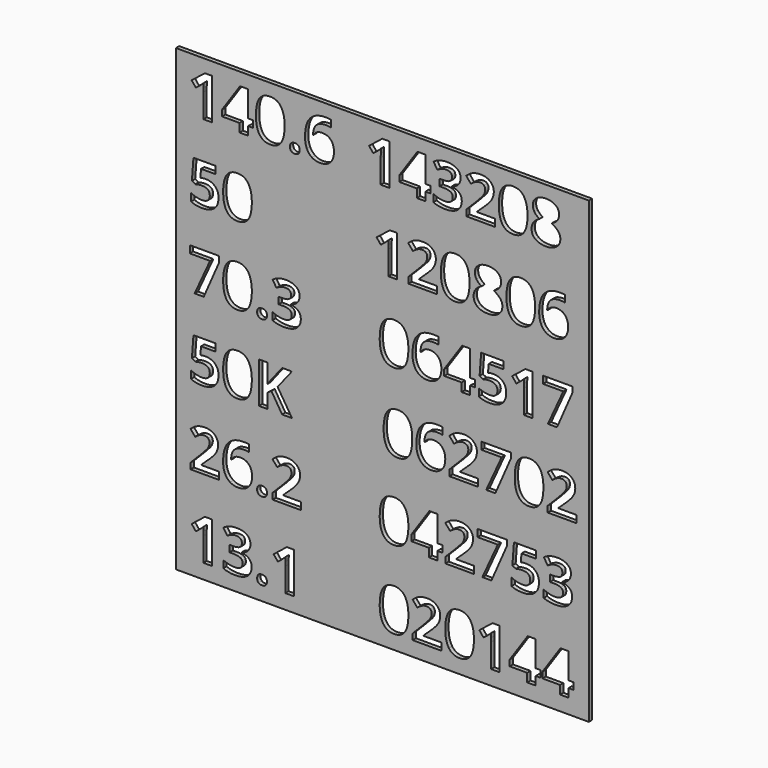
from build123d import *

# Parameters (mm, degrees)
F0_W     = 99.8563368056
F0_H     = 111
F1_DEPTH = 1


with BuildPart() as f1:
    # F0 (on Front) → F1 (new body)
    with BuildSketch(Plane.XZ):
        with Locations((1.7441204268, -63.4162358642)):
            Rectangle(F0_W, F0_H)
        with BuildLine():
            Line((-39.4462007537, -105.4453157253), (-39.4462007537, -115.3606803086))
            Line((-39.4462007537, -115.3606803086), (-41.5425549204, -115.3606803086))
            Line((-41.5425549204, -115.3606803086), (-41.5425549204, -109.6228330864))
            Line((-41.5425549204, -109.6228330864), (-41.5208535315, -108.6809928086))
            Line((-41.5208535315, -108.6809928086), (-41.4883014482, -107.6501768364))
            add(Edge.make_bspline(
                [(-41.4883014482, -107.6501768364), (-42.0091347815, -108.1710101697), (-42.2131278371, -108.3337705864)],
                knots=[0, 0, 0, 1, 1, 1], degree=2))
            Line((-42.2131278371, -108.3337705864), (-43.3524507537, -109.2495691975))
            Line((-43.3524507537, -109.2495691975), (-44.363735476, -107.9887185031))
            Line((-44.363735476, -107.9887185031), (-41.1692910315, -105.4453157253))
            Line((-41.1692910315, -105.4453157253), (-39.4462007537, -105.4453157253))
        make_face(mode=Mode.SUBTRACT)
        with BuildLine():
            add(Edge.make_bspline(
                [(-28.2233274899, -115.2413226697), (-28.5347424204, -114.9396733642), (-28.5347424204, -114.3906282253)],
                knots=[0, 0, 0, 1, 1, 1], degree=2))
            add(Edge.make_bspline(
                [(-28.5347424204, -114.3906282253), (-28.5347424204, -113.8220518364), (-28.2298379065, -113.5301681558)],
                knots=[0, 0, 0, 1, 1, 1], degree=2))
            add(Edge.make_bspline(
                [(-28.2298379065, -113.5301681558), (-27.9249333926, -113.2382844753), (-27.3411660315, -113.2382844753)],
                knots=[0, 0, 0, 1, 1, 1], degree=2))
            add(Edge.make_bspline(
                [(-27.3411660315, -113.2382844753), (-26.7791000593, -113.2382844753), (-26.4709403371, -113.5366785725)],
                knots=[0, 0, 0, 1, 1, 1], degree=2))
            add(Edge.make_bspline(
                [(-26.4709403371, -113.5366785725), (-26.1627806149, -113.8350726697), (-26.1627806149, -114.3906282253)],
                knots=[0, 0, 0, 1, 1, 1], degree=2))
            add(Edge.make_bspline(
                [(-26.1627806149, -114.3906282253), (-26.1627806149, -114.9266525308), (-26.4741955454, -115.2348122531)],
                knots=[0, 0, 0, 1, 1, 1], degree=2))
            add(Edge.make_bspline(
                [(-26.4741955454, -115.2348122531), (-26.785610476, -115.5429719753), (-27.3411660315, -115.5429719753)],
                knots=[0, 0, 0, 1, 1, 1], degree=2))
            add(Edge.make_bspline(
                [(-27.3411660315, -115.5429719753), (-27.9119125593, -115.5429719753), (-28.2233274899, -115.2413226697)],
                knots=[0, 0, 0, 1, 1, 1], degree=2))
        make_face(mode=Mode.SUBTRACT)
        with BuildLine():
            add(Edge.make_bspline(
                [(-31.0477632537, -105.9281716281), (-30.1558361704, -106.5520865586), (-30.1558361704, -107.6631976697)],
                knots=[0, 0, 0, 1, 1, 1], degree=2))
            add(Edge.make_bspline(
                [(-30.1558361704, -107.6631976697), (-30.1558361704, -108.5920171142), (-30.7189872121, -109.2430587808)],
                knots=[0, 0, 0, 1, 1, 1], degree=2))
            add(Edge.make_bspline(
                [(-30.7189872121, -109.2430587808), (-31.2821382537, -109.8941004475), (-32.2999333926, -110.1393261419)],
                knots=[0, 0, 0, 1, 1, 1], degree=2))
            Line((-32.2999333926, -110.1393261419), (-32.2999333926, -110.1783886419))
            add(Edge.make_bspline(
                [(-32.2999333926, -110.1783886419), (-31.0976764482, -110.3281282253), (-30.4813570037, -110.9086403781)],
                knots=[0, 0, 0, 1, 1, 1], degree=2))
            add(Edge.make_bspline(
                [(-30.4813570037, -110.9086403781), (-29.8650375593, -111.4891525308), (-29.8650375593, -112.4722254475)],
                knots=[0, 0, 0, 1, 1, 1], degree=2))
            add(Edge.make_bspline(
                [(-29.8650375593, -112.4722254475), (-29.8650375593, -113.9023469753), (-30.9023639482, -114.6998730169)],
                knots=[0, 0, 0, 1, 1, 1], degree=2))
            add(Edge.make_bspline(
                [(-30.9023639482, -114.6998730169), (-31.9396903371, -115.4973990586), (-33.8646035315, -115.4973990586)],
                knots=[0, 0, 0, 1, 1, 1], degree=2))
            add(Edge.make_bspline(
                [(-33.8646035315, -115.4973990586), (-35.4791868649, -115.4973990586), (-36.727016726, -114.9613747531)],
                knots=[0, 0, 0, 1, 1, 1], degree=2))
            Line((-36.727016726, -114.9613747531), (-36.727016726, -113.1775205864))
            add(Edge.make_bspline(
                [(-36.727016726, -113.1775205864), (-36.1519299204, -113.4683191975), (-35.4596556149, -113.6516959336)],
                knots=[0, 0, 0, 1, 1, 1], degree=2))
            add(Edge.make_bspline(
                [(-35.4596556149, -113.6516959336), (-34.7673813093, -113.8350726697), (-34.090297976, -113.8350726697)],
                knots=[0, 0, 0, 1, 1, 1], degree=2))
            add(Edge.make_bspline(
                [(-34.090297976, -113.8350726697), (-33.0508014482, -113.8350726697), (-32.5560097815, -113.4824251003)],
                knots=[0, 0, 0, 1, 1, 1], degree=2))
            add(Edge.make_bspline(
                [(-32.5560097815, -113.4824251003), (-32.0612181149, -113.1297775308), (-32.0612181149, -112.3485275308)],
                knots=[0, 0, 0, 1, 1, 1], degree=2))
            add(Edge.make_bspline(
                [(-32.0612181149, -112.3485275308), (-32.0612181149, -111.6519129475), (-32.6308795732, -111.3600292669)],
                knots=[0, 0, 0, 1, 1, 1], degree=2))
            add(Edge.make_bspline(
                [(-32.6308795732, -111.3600292669), (-33.2005410315, -111.0681455864), (-34.4483708926, -111.0681455864)],
                knots=[0, 0, 0, 1, 1, 1], degree=2))
            Line((-34.4483708926, -111.0681455864), (-35.2014090871, -111.0681455864))
            Line((-35.2014090871, -111.0681455864), (-35.2014090871, -109.4600726697))
            Line((-35.2014090871, -109.4600726697), (-34.4353500593, -109.4600726697))
            add(Edge.make_bspline(
                [(-34.4353500593, -109.4600726697), (-33.2830063093, -109.4600726697), (-32.7502372121, -109.1584233642)],
                knots=[0, 0, 0, 1, 1, 1], degree=2))
            add(Edge.make_bspline(
                [(-32.7502372121, -109.1584233642), (-32.2174681149, -108.8567740586), (-32.2174681149, -108.1254372531)],
                knots=[0, 0, 0, 1, 1, 1], degree=2))
            add(Edge.make_bspline(
                [(-32.2174681149, -108.1254372531), (-32.2174681149, -106.9991351697), (-33.6280583926, -106.9991351697)],
                knots=[0, 0, 0, 1, 1, 1], degree=2))
            add(Edge.make_bspline(
                [(-33.6280583926, -106.9991351697), (-34.1163396426, -106.9991351697), (-34.6219820037, -107.1618955864)],
                knots=[0, 0, 0, 1, 1, 1], degree=2))
            add(Edge.make_bspline(
                [(-34.6219820037, -107.1618955864), (-35.1276243649, -107.3246560031), (-35.7439438093, -107.7239615586)],
                knots=[0, 0, 0, 1, 1, 1], degree=2))
            Line((-35.7439438093, -107.7239615586), (-36.7139958926, -106.2808191975))
            add(Edge.make_bspline(
                [(-36.7139958926, -106.2808191975), (-35.3576590871, -105.3042566975), (-33.4783188093, -105.3042566975)],
                knots=[0, 0, 0, 1, 1, 1], degree=2))
            add(Edge.make_bspline(
                [(-33.4783188093, -105.3042566975), (-31.9396903371, -105.3042566975), (-31.0477632537, -105.9281716281)],
                knots=[0, 0, 0, 1, 1, 1], degree=2))
        make_face(mode=Mode.SUBTRACT)
        with BuildLine():
            Line((-37.6970688093, -94.7074685031), (-37.6970688093, -96.4717914197))
            Line((-37.6970688093, -96.4717914197), (-44.6284924204, -96.4717914197))
            Line((-44.6284924204, -96.4717914197), (-44.6284924204, -95.0134580864))
            Line((-44.6284924204, -95.0134580864), (-42.1393431149, -92.4982671142))
            add(Edge.make_bspline(
                [(-42.1393431149, -92.4982671142), (-41.0325722815, -91.3654546142), (-40.6940306149, -90.9281716281)],
                knots=[0, 0, 0, 1, 1, 1], degree=2))
            add(Edge.make_bspline(
                [(-40.6940306149, -90.9281716281), (-40.3554889482, -90.4908886419), (-40.2057493649, -90.1176247531)],
                knots=[0, 0, 0, 1, 1, 1], degree=2))
            add(Edge.make_bspline(
                [(-40.2057493649, -90.1176247531), (-40.0560097815, -89.7443608642), (-40.0560097815, -89.3450553086)],
                knots=[0, 0, 0, 1, 1, 1], degree=2))
            add(Edge.make_bspline(
                [(-40.0560097815, -89.3450553086), (-40.0560097815, -88.7482671142), (-40.3858708926, -88.4563834336)],
                knots=[0, 0, 0, 1, 1, 1], degree=2))
            add(Edge.make_bspline(
                [(-40.3858708926, -88.4563834336), (-40.7157320037, -88.1644997531), (-41.2647771426, -88.1644997531)],
                knots=[0, 0, 0, 1, 1, 1], degree=2))
            add(Edge.make_bspline(
                [(-41.2647771426, -88.1644997531), (-41.8398639482, -88.1644997531), (-42.3823986704, -88.4292566975)],
                knots=[0, 0, 0, 1, 1, 1], degree=2))
            add(Edge.make_bspline(
                [(-42.3823986704, -88.4292566975), (-42.9249333926, -88.6940136419), (-43.5152111704, -89.1822948919)],
                knots=[0, 0, 0, 1, 1, 1], degree=2))
            Line((-43.5152111704, -89.1822948919), (-44.6545340871, -87.8324685031))
            add(Edge.make_bspline(
                [(-44.6545340871, -87.8324685031), (-43.9231972815, -87.2074685031), (-43.4414264482, -86.9503070447)],
                knots=[0, 0, 0, 1, 1, 1], degree=2))
            add(Edge.make_bspline(
                [(-43.4414264482, -86.9503070447), (-42.9596556149, -86.6931455864), (-42.3899941565, -86.5542566975)],
                knots=[0, 0, 0, 1, 1, 1], degree=2))
            add(Edge.make_bspline(
                [(-42.3899941565, -86.5542566975), (-41.8203326982, -86.4153678086), (-41.1150375593, -86.4153678086)],
                knots=[0, 0, 0, 1, 1, 1], degree=2))
            add(Edge.make_bspline(
                [(-41.1150375593, -86.4153678086), (-40.1862181149, -86.4153678086), (-39.4744125593, -86.7539094753)],
                knots=[0, 0, 0, 1, 1, 1], degree=2))
            add(Edge.make_bspline(
                [(-39.4744125593, -86.7539094753), (-38.7626070037, -87.0924511419), (-38.3687267954, -87.7033452392)],
                knots=[0, 0, 0, 1, 1, 1], degree=2))
            add(Edge.make_bspline(
                [(-38.3687267954, -87.7033452392), (-37.9748465871, -88.3142393364), (-37.9748465871, -89.0998296142)],
                knots=[0, 0, 0, 1, 1, 1], degree=2))
            add(Edge.make_bspline(
                [(-37.9748465871, -89.0998296142), (-37.9748465871, -89.7855935031), (-38.2157320037, -90.3856369058)],
                knots=[0, 0, 0, 1, 1, 1], degree=2))
            add(Edge.make_bspline(
                [(-38.2157320037, -90.3856369058), (-38.4566174204, -90.9856803086), (-38.9622597815, -91.6161056558)],
                knots=[0, 0, 0, 1, 1, 1], degree=2))
            add(Edge.make_bspline(
                [(-38.9622597815, -91.6161056558), (-39.4679021426, -92.2465310031), (-40.7417736704, -93.4140657253)],
                knots=[0, 0, 0, 1, 1, 1], degree=2))
            Line((-40.7417736704, -93.4140657253), (-42.0178153371, -94.6141525308))
            Line((-42.0178153371, -94.6141525308), (-42.0178153371, -94.7074685031))
            Line((-42.0178153371, -94.7074685031), (-37.6970688093, -94.7074685031))
        make_face(mode=Mode.SUBTRACT)
        with BuildLine():
            add(Edge.make_bspline(
                [(-36.3244559621, -94.6141525308), (-36.7682493649, -93.6375900308), (-36.7682493649, -92.2595518364)],
                knots=[0, 0, 0, 1, 1, 1], degree=2))
            add(Edge.make_bspline(
                [(-36.7682493649, -92.2595518364), (-36.7682493649, -89.3168435031), (-35.5236747121, -87.8791264892)],
                knots=[0, 0, 0, 1, 1, 1], degree=2))
            add(Edge.make_bspline(
                [(-35.5236747121, -87.8791264892), (-34.2791000593, -86.4414094753), (-31.7964611704, -86.4414094753)],
                knots=[0, 0, 0, 1, 1, 1], degree=2))
            add(Edge.make_bspline(
                [(-31.7964611704, -86.4414094753), (-30.9501070037, -86.4414094753), (-30.4683361704, -86.5434060031)],
                knots=[0, 0, 0, 1, 1, 1], degree=2))
            Line((-30.4683361704, -86.5434060031), (-30.4683361704, -88.2187532253))
            add(Edge.make_bspline(
                [(-30.4683361704, -88.2187532253), (-31.0716347815, -88.0820344753), (-31.6619125593, -88.0820344753)],
                knots=[0, 0, 0, 1, 1, 1], degree=2))
            add(Edge.make_bspline(
                [(-31.6619125593, -88.0820344753), (-32.7404715871, -88.0820344753), (-33.4218951982, -88.4075553086)],
                knots=[0, 0, 0, 1, 1, 1], degree=2))
            add(Edge.make_bspline(
                [(-33.4218951982, -88.4075553086), (-34.1033188093, -88.7330761419), (-34.441860476, -89.3710969753)],
                knots=[0, 0, 0, 1, 1, 1], degree=2))
            add(Edge.make_bspline(
                [(-34.441860476, -89.3710969753), (-34.7804021426, -90.0091178086), (-34.8411660315, -91.1809928086)],
                knots=[0, 0, 0, 1, 1, 1], degree=2))
            Line((-34.8411660315, -91.1809928086), (-34.754360476, -91.1809928086))
            add(Edge.make_bspline(
                [(-34.754360476, -91.1809928086), (-34.0816174204, -90.0286490586), (-32.6037528371, -90.0286490586)],
                knots=[0, 0, 0, 1, 1, 1], degree=2))
            add(Edge.make_bspline(
                [(-32.6037528371, -90.0286490586), (-31.2756278371, -90.0286490586), (-30.5225896426, -90.8630674614)],
                knots=[0, 0, 0, 1, 1, 1], degree=2))
            add(Edge.make_bspline(
                [(-30.5225896426, -90.8630674614), (-29.7695514482, -91.6974858642), (-29.7695514482, -93.1688400308)],
                knots=[0, 0, 0, 1, 1, 1], degree=2))
            add(Edge.make_bspline(
                [(-29.7695514482, -93.1688400308), (-29.7695514482, -94.7552115586), (-30.6647337399, -95.6818608642)],
                knots=[0, 0, 0, 1, 1, 1], degree=2))
            add(Edge.make_bspline(
                [(-30.6647337399, -95.6818608642), (-31.5599160315, -96.6085101697), (-33.1462875593, -96.6085101697)],
                knots=[0, 0, 0, 1, 1, 1], degree=2))
            add(Edge.make_bspline(
                [(-33.1462875593, -96.6085101697), (-34.2443778371, -96.6085101697), (-35.0625201982, -96.0996126003)],
                knots=[0, 0, 0, 1, 1, 1], degree=2))
            add(Edge.make_bspline(
                [(-35.0625201982, -96.0996126003), (-35.8806625593, -95.5907150308), (-36.3244559621, -94.6141525308)],
                knots=[0, 0, 0, 1, 1, 1], degree=2))
        make_face(mode=Mode.SUBTRACT)
        with BuildLine():
            add(Edge.make_bspline(
                [(-28.2233274899, -96.3524337808), (-28.5347424204, -96.0507844753), (-28.5347424204, -95.5017393364)],
                knots=[0, 0, 0, 1, 1, 1], degree=2))
            add(Edge.make_bspline(
                [(-28.5347424204, -95.5017393364), (-28.5347424204, -94.9331629475), (-28.2298379065, -94.6412792669)],
                knots=[0, 0, 0, 1, 1, 1], degree=2))
            add(Edge.make_bspline(
                [(-28.2298379065, -94.6412792669), (-27.9249333926, -94.3493955864), (-27.3411660315, -94.3493955864)],
                knots=[0, 0, 0, 1, 1, 1], degree=2))
            add(Edge.make_bspline(
                [(-27.3411660315, -94.3493955864), (-26.7791000593, -94.3493955864), (-26.4709403371, -94.6477896836)],
                knots=[0, 0, 0, 1, 1, 1], degree=2))
            add(Edge.make_bspline(
                [(-26.4709403371, -94.6477896836), (-26.1627806149, -94.9461837808), (-26.1627806149, -95.5017393364)],
                knots=[0, 0, 0, 1, 1, 1], degree=2))
            add(Edge.make_bspline(
                [(-26.1627806149, -95.5017393364), (-26.1627806149, -96.0377636419), (-26.4741955454, -96.3459233642)],
                knots=[0, 0, 0, 1, 1, 1], degree=2))
            add(Edge.make_bspline(
                [(-26.4741955454, -96.3459233642), (-26.785610476, -96.6540830864), (-27.3411660315, -96.6540830864)],
                knots=[0, 0, 0, 1, 1, 1], degree=2))
            add(Edge.make_bspline(
                [(-27.3411660315, -96.6540830864), (-27.9119125593, -96.6540830864), (-28.2233274899, -96.3524337808)],
                knots=[0, 0, 0, 1, 1, 1], degree=2))
        make_face(mode=Mode.SUBTRACT)
        with BuildLine():
            Line((-19.6306625593, -105.4453157253), (-19.6306625593, -115.3606803086))
            Line((-19.6306625593, -115.3606803086), (-21.727016726, -115.3606803086))
            Line((-21.727016726, -115.3606803086), (-21.727016726, -109.6228330864))
            Line((-21.727016726, -109.6228330864), (-21.7053153371, -108.6809928086))
            Line((-21.7053153371, -108.6809928086), (-21.6727632537, -107.6501768364))
            add(Edge.make_bspline(
                [(-21.6727632537, -107.6501768364), (-22.1935965871, -108.1710101697), (-22.3975896426, -108.3337705864)],
                knots=[0, 0, 0, 1, 1, 1], degree=2))
            Line((-22.3975896426, -108.3337705864), (-23.5369125593, -109.2495691975))
            Line((-23.5369125593, -109.2495691975), (-24.5481972815, -107.9887185031))
            Line((-24.5481972815, -107.9887185031), (-21.3537528371, -105.4453157253))
            Line((-21.3537528371, -105.4453157253), (-19.6306625593, -105.4453157253))
        make_face(mode=Mode.SUBTRACT)
        with BuildLine():
            Line((-17.8815306149, -94.7074685031), (-17.8815306149, -96.4717914197))
            Line((-17.8815306149, -96.4717914197), (-24.812954226, -96.4717914197))
            Line((-24.812954226, -96.4717914197), (-24.812954226, -95.0134580864))
            Line((-24.812954226, -95.0134580864), (-22.3238049204, -92.4982671142))
            add(Edge.make_bspline(
                [(-22.3238049204, -92.4982671142), (-21.2170340871, -91.3654546142), (-20.8784924204, -90.9281716281)],
                knots=[0, 0, 0, 1, 1, 1], degree=2))
            add(Edge.make_bspline(
                [(-20.8784924204, -90.9281716281), (-20.5399507537, -90.4908886419), (-20.3902111704, -90.1176247531)],
                knots=[0, 0, 0, 1, 1, 1], degree=2))
            add(Edge.make_bspline(
                [(-20.3902111704, -90.1176247531), (-20.2404715871, -89.7443608642), (-20.2404715871, -89.3450553086)],
                knots=[0, 0, 0, 1, 1, 1], degree=2))
            add(Edge.make_bspline(
                [(-20.2404715871, -89.3450553086), (-20.2404715871, -88.7482671142), (-20.5703326982, -88.4563834336)],
                knots=[0, 0, 0, 1, 1, 1], degree=2))
            add(Edge.make_bspline(
                [(-20.5703326982, -88.4563834336), (-20.9001938093, -88.1644997531), (-21.4492389482, -88.1644997531)],
                knots=[0, 0, 0, 1, 1, 1], degree=2))
            add(Edge.make_bspline(
                [(-21.4492389482, -88.1644997531), (-22.0243257537, -88.1644997531), (-22.566860476, -88.4292566975)],
                knots=[0, 0, 0, 1, 1, 1], degree=2))
            add(Edge.make_bspline(
                [(-22.566860476, -88.4292566975), (-23.1093951982, -88.6940136419), (-23.699672976, -89.1822948919)],
                knots=[0, 0, 0, 1, 1, 1], degree=2))
            Line((-23.699672976, -89.1822948919), (-24.8389958926, -87.8324685031))
            add(Edge.make_bspline(
                [(-24.8389958926, -87.8324685031), (-24.1076590871, -87.2074685031), (-23.6258882537, -86.9503070447)],
                knots=[0, 0, 0, 1, 1, 1], degree=2))
            add(Edge.make_bspline(
                [(-23.6258882537, -86.9503070447), (-23.1441174204, -86.6931455864), (-22.5744559621, -86.5542566975)],
                knots=[0, 0, 0, 1, 1, 1], degree=2))
            add(Edge.make_bspline(
                [(-22.5744559621, -86.5542566975), (-22.0047945037, -86.4153678086), (-21.2994993649, -86.4153678086)],
                knots=[0, 0, 0, 1, 1, 1], degree=2))
            add(Edge.make_bspline(
                [(-21.2994993649, -86.4153678086), (-20.3706799204, -86.4153678086), (-19.6588743649, -86.7539094753)],
                knots=[0, 0, 0, 1, 1, 1], degree=2))
            add(Edge.make_bspline(
                [(-19.6588743649, -86.7539094753), (-18.9470688093, -87.0924511419), (-18.553188601, -87.7033452392)],
                knots=[0, 0, 0, 1, 1, 1], degree=2))
            add(Edge.make_bspline(
                [(-18.553188601, -87.7033452392), (-18.1593083926, -88.3142393364), (-18.1593083926, -89.0998296142)],
                knots=[0, 0, 0, 1, 1, 1], degree=2))
            add(Edge.make_bspline(
                [(-18.1593083926, -89.0998296142), (-18.1593083926, -89.7855935031), (-18.4001938093, -90.3856369058)],
                knots=[0, 0, 0, 1, 1, 1], degree=2))
            add(Edge.make_bspline(
                [(-18.4001938093, -90.3856369058), (-18.641079226, -90.9856803086), (-19.1467215871, -91.6161056558)],
                knots=[0, 0, 0, 1, 1, 1], degree=2))
            add(Edge.make_bspline(
                [(-19.1467215871, -91.6161056558), (-19.6523639482, -92.2465310031), (-20.926235476, -93.4140657253)],
                knots=[0, 0, 0, 1, 1, 1], degree=2))
            Line((-20.926235476, -93.4140657253), (-22.2022771426, -94.6141525308))
            Line((-22.2022771426, -94.6141525308), (-22.2022771426, -94.7074685031))
            Line((-22.2022771426, -94.7074685031), (-17.8815306149, -94.7074685031))
        make_face(mode=Mode.SUBTRACT)
        with BuildLine():
            add(Edge.make_bspline(
                [(-42.0438570037, -71.3437532253), (-41.629360476, -71.2482671142), (-41.0195514482, -71.2482671142)],
                knots=[0, 0, 0, 1, 1, 1], degree=2))
            add(Edge.make_bspline(
                [(-41.0195514482, -71.2482671142), (-39.5829195037, -71.2482671142), (-38.7311399899, -72.0555587808)],
                knots=[0, 0, 0, 1, 1, 1], degree=2))
            add(Edge.make_bspline(
                [(-38.7311399899, -72.0555587808), (-37.879360476, -72.8628504475), (-37.879360476, -74.2669303086)],
                knots=[0, 0, 0, 1, 1, 1], degree=2))
            add(Edge.make_bspline(
                [(-37.879360476, -74.2669303086), (-37.879360476, -75.9270865586), (-38.9036660315, -76.8233539197)],
                knots=[0, 0, 0, 1, 1, 1], degree=2))
            add(Edge.make_bspline(
                [(-38.9036660315, -76.8233539197), (-39.9279715871, -77.7196212808), (-41.8333535315, -77.7196212808)],
                knots=[0, 0, 0, 1, 1, 1], degree=2))
            add(Edge.make_bspline(
                [(-41.8333535315, -77.7196212808), (-43.4891695037, -77.7196212808), (-44.5047945037, -77.1835969753)],
                knots=[0, 0, 0, 1, 1, 1], degree=2))
            Line((-44.5047945037, -77.1835969753), (-44.5047945037, -75.3715310031))
            add(Edge.make_bspline(
                [(-44.5047945037, -75.3715310031), (-43.9709403371, -75.6558191975), (-43.2580497121, -75.8359407253)],
                knots=[0, 0, 0, 1, 1, 1], degree=2))
            add(Edge.make_bspline(
                [(-43.2580497121, -75.8359407253), (-42.5451590871, -76.0160622531), (-41.9093083926, -76.0160622531)],
                knots=[0, 0, 0, 1, 1, 1], degree=2))
            add(Edge.make_bspline(
                [(-41.9093083926, -76.0160622531), (-39.988735476, -76.0160622531), (-39.988735476, -74.4427115586)],
                knots=[0, 0, 0, 1, 1, 1], degree=2))
            add(Edge.make_bspline(
                [(-39.988735476, -74.4427115586), (-39.988735476, -72.9431455864), (-41.9765826982, -72.9431455864)],
                knots=[0, 0, 0, 1, 1, 1], degree=2))
            add(Edge.make_bspline(
                [(-41.9765826982, -72.9431455864), (-42.3346556149, -72.9431455864), (-42.7686833926, -73.0147601697)],
                knots=[0, 0, 0, 1, 1, 1], degree=2))
            add(Edge.make_bspline(
                [(-42.7686833926, -73.0147601697), (-43.2027111704, -73.0863747531), (-43.4739785315, -73.1688400308)],
                knots=[0, 0, 0, 1, 1, 1], degree=2))
            Line((-43.4739785315, -73.1688400308), (-44.3094820037, -72.7196212808))
            Line((-44.3094820037, -72.7196212808), (-43.9362181149, -67.6675379475))
            Line((-43.9362181149, -67.6675379475), (-38.5586139482, -67.6675379475))
            Line((-38.5586139482, -67.6675379475), (-38.5586139482, -69.4448816975))
            Line((-38.5586139482, -69.4448816975), (-42.098110476, -69.4448816975))
            Line((-42.098110476, -69.4448816975), (-42.2804021426, -71.3914962808))
            Line((-42.2804021426, -71.3914962808), (-42.0438570037, -71.3437532253))
        make_face(mode=Mode.SUBTRACT)
        with BuildLine():
            add(Edge.make_bspline(
                [(-30.701626101, -68.8133712808), (-29.8238049204, -70.1154546142), (-29.8238049204, -72.6263053086)],
                knots=[0, 0, 0, 1, 1, 1], degree=2))
            add(Edge.make_bspline(
                [(-29.8238049204, -72.6263053086), (-29.8238049204, -75.2217914197), (-30.6744993649, -76.4707063503)],
                knots=[0, 0, 0, 1, 1, 1], degree=2))
            add(Edge.make_bspline(
                [(-30.6744993649, -76.4707063503), (-31.5251938093, -77.7196212808), (-33.2960271426, -77.7196212808)],
                knots=[0, 0, 0, 1, 1, 1], degree=2))
            add(Edge.make_bspline(
                [(-33.2960271426, -77.7196212808), (-35.0126070037, -77.7196212808), (-35.8839177676, -76.4305587808)],
                knots=[0, 0, 0, 1, 1, 1], degree=2))
            add(Edge.make_bspline(
                [(-35.8839177676, -76.4305587808), (-36.7552285315, -75.1414962808), (-36.7552285315, -72.6263053086)],
                knots=[0, 0, 0, 1, 1, 1], degree=2))
            add(Edge.make_bspline(
                [(-36.7552285315, -72.6263053086), (-36.7552285315, -70.0004372531), (-35.906704226, -68.7558626003)],
                knots=[0, 0, 0, 1, 1, 1], degree=2))
            add(Edge.make_bspline(
                [(-35.906704226, -68.7558626003), (-35.0581799204, -67.5112879475), (-33.2960271426, -67.5112879475)],
                knots=[0, 0, 0, 1, 1, 1], degree=2))
            add(Edge.make_bspline(
                [(-33.2960271426, -67.5112879475), (-31.5794472815, -67.5112879475), (-30.701626101, -68.8133712808)],
                knots=[0, 0, 0, 1, 1, 1], degree=2))
        make_face(mode=Mode.SUBTRACT)
        Polygon((-23.5911660315, -72.0555587808), (-20.105922976, -77.5829025308), (-22.4930757537, -77.5829025308), (-25.0907320037, -73.4053851697), (-25.9783188093, -74.0434060031), (-25.9783188093, -77.5829025308), (-28.0811833926, -77.5829025308), (-28.0811833926, -67.6675379475), (-25.9783188093, -67.6675379475), (-25.9783188093, -72.2052983642), (-25.1514958926, -71.0377636419), (-22.4648639482, -67.6675379475), (-20.1319646426, -67.6675379475), align=None, mode=Mode.SUBTRACT)
        with BuildLine():
            add(Edge.make_bspline(
                [(7.1586169546, -106.5911490586), (8.0364381351, -107.8932323919), (8.0364381351, -110.4040830864)],
                knots=[0, 0, 0, 1, 1, 1], degree=2))
            add(Edge.make_bspline(
                [(8.0364381351, -110.4040830864), (8.0364381351, -112.9995691975), (7.1857436907, -114.2484841281)],
                knots=[0, 0, 0, 1, 1, 1], degree=2))
            add(Edge.make_bspline(
                [(7.1857436907, -114.2484841281), (6.3350492463, -115.4973990586), (4.5642159129, -115.4973990586)],
                knots=[0, 0, 0, 1, 1, 1], degree=2))
            add(Edge.make_bspline(
                [(4.5642159129, -115.4973990586), (2.8476360518, -115.4973990586), (1.9763252879, -114.2083365586)],
                knots=[0, 0, 0, 1, 1, 1], degree=2))
            add(Edge.make_bspline(
                [(1.9763252879, -114.2083365586), (1.105014524, -112.9192740586), (1.105014524, -110.4040830864)],
                knots=[0, 0, 0, 1, 1, 1], degree=2))
            add(Edge.make_bspline(
                [(1.105014524, -110.4040830864), (1.105014524, -107.7782150308), (1.9535388296, -106.5336403781)],
                knots=[0, 0, 0, 1, 1, 1], degree=2))
            add(Edge.make_bspline(
                [(1.9535388296, -106.5336403781), (2.8020631351, -105.2890657253), (4.5642159129, -105.2890657253)],
                knots=[0, 0, 0, 1, 1, 1], degree=2))
            add(Edge.make_bspline(
                [(4.5642159129, -105.2890657253), (6.280795774, -105.2890657253), (7.1586169546, -106.5911490586)],
                knots=[0, 0, 0, 1, 1, 1], degree=2))
        make_face(mode=Mode.SUBTRACT)
        with BuildLine():
            Line((16.0182089685, -113.5963573919), (16.0182089685, -115.3606803086))
            Line((16.0182089685, -115.3606803086), (9.0867853574, -115.3606803086))
            Line((9.0867853574, -115.3606803086), (9.0867853574, -113.9023469753))
            Line((9.0867853574, -113.9023469753), (11.5759346629, -111.3871560031))
            add(Edge.make_bspline(
                [(11.5759346629, -111.3871560031), (12.6827054963, -110.2543435031), (13.0212471629, -109.8170605169)],
                knots=[0, 0, 0, 1, 1, 1], degree=2))
            add(Edge.make_bspline(
                [(13.0212471629, -109.8170605169), (13.3597888296, -109.3797775308), (13.5095284129, -109.0065136419)],
                knots=[0, 0, 0, 1, 1, 1], degree=2))
            add(Edge.make_bspline(
                [(13.5095284129, -109.0065136419), (13.6592679963, -108.6332497531), (13.6592679963, -108.2339441975)],
                knots=[0, 0, 0, 1, 1, 1], degree=2))
            add(Edge.make_bspline(
                [(13.6592679963, -108.2339441975), (13.6592679963, -107.6371560031), (13.3294068851, -107.3452723225)],
                knots=[0, 0, 0, 1, 1, 1], degree=2))
            add(Edge.make_bspline(
                [(13.3294068851, -107.3452723225), (12.999545774, -107.0533886419), (12.4505006351, -107.0533886419)],
                knots=[0, 0, 0, 1, 1, 1], degree=2))
            add(Edge.make_bspline(
                [(12.4505006351, -107.0533886419), (11.8754138296, -107.0533886419), (11.3328791074, -107.3181455864)],
                knots=[0, 0, 0, 1, 1, 1], degree=2))
            add(Edge.make_bspline(
                [(11.3328791074, -107.3181455864), (10.7903443851, -107.5829025308), (10.2000666074, -108.0711837808)],
                knots=[0, 0, 0, 1, 1, 1], degree=2))
            Line((10.2000666074, -108.0711837808), (9.0607436907, -106.7213573919))
            add(Edge.make_bspline(
                [(9.0607436907, -106.7213573919), (9.7920804963, -106.0963573919), (10.2738513296, -105.8391959336)],
                knots=[0, 0, 0, 1, 1, 1], degree=2))
            add(Edge.make_bspline(
                [(10.2738513296, -105.8391959336), (10.7556221629, -105.5820344753), (11.3252836213, -105.4431455864)],
                knots=[0, 0, 0, 1, 1, 1], degree=2))
            add(Edge.make_bspline(
                [(11.3252836213, -105.4431455864), (11.8949450796, -105.3042566975), (12.6002402185, -105.3042566975)],
                knots=[0, 0, 0, 1, 1, 1], degree=2))
            add(Edge.make_bspline(
                [(12.6002402185, -105.3042566975), (13.5290596629, -105.3042566975), (14.2408652185, -105.6427983642)],
                knots=[0, 0, 0, 1, 1, 1], degree=2))
            add(Edge.make_bspline(
                [(14.2408652185, -105.6427983642), (14.952670774, -105.9813400308), (15.3465509824, -106.5922341281)],
                knots=[0, 0, 0, 1, 1, 1], degree=2))
            add(Edge.make_bspline(
                [(15.3465509824, -106.5922341281), (15.7404311907, -107.2031282253), (15.7404311907, -107.9887185031)],
                knots=[0, 0, 0, 1, 1, 1], degree=2))
            add(Edge.make_bspline(
                [(15.7404311907, -107.9887185031), (15.7404311907, -108.6744823919), (15.499545774, -109.2745257947)],
                knots=[0, 0, 0, 1, 1, 1], degree=2))
            add(Edge.make_bspline(
                [(15.499545774, -109.2745257947), (15.2586603574, -109.8745691975), (14.7530179963, -110.5049945447)],
                knots=[0, 0, 0, 1, 1, 1], degree=2))
            add(Edge.make_bspline(
                [(14.7530179963, -110.5049945447), (14.2473756351, -111.1354198919), (12.9735041074, -112.3029546142)],
                knots=[0, 0, 0, 1, 1, 1], degree=2))
            Line((12.9735041074, -112.3029546142), (11.6974624407, -113.5030414197))
            Line((11.6974624407, -113.5030414197), (11.6974624407, -113.5963573919))
            Line((11.6974624407, -113.5963573919), (16.0182089685, -113.5963573919))
        make_face(mode=Mode.SUBTRACT)
        with BuildLine():
            add(Edge.make_bspline(
                [(23.0136516768, -106.5911490586), (23.8914728574, -107.8932323919), (23.8914728574, -110.4040830864)],
                knots=[0, 0, 0, 1, 1, 1], degree=2))
            add(Edge.make_bspline(
                [(23.8914728574, -110.4040830864), (23.8914728574, -112.9995691975), (23.0407784129, -114.2484841281)],
                knots=[0, 0, 0, 1, 1, 1], degree=2))
            add(Edge.make_bspline(
                [(23.0407784129, -114.2484841281), (22.1900839685, -115.4973990586), (20.4192506351, -115.4973990586)],
                knots=[0, 0, 0, 1, 1, 1], degree=2))
            add(Edge.make_bspline(
                [(20.4192506351, -115.4973990586), (18.702670774, -115.4973990586), (17.8313600101, -114.2083365586)],
                knots=[0, 0, 0, 1, 1, 1], degree=2))
            add(Edge.make_bspline(
                [(17.8313600101, -114.2083365586), (16.9600492463, -112.9192740586), (16.9600492463, -110.4040830864)],
                knots=[0, 0, 0, 1, 1, 1], degree=2))
            add(Edge.make_bspline(
                [(16.9600492463, -110.4040830864), (16.9600492463, -107.7782150308), (17.8085735518, -106.5336403781)],
                knots=[0, 0, 0, 1, 1, 1], degree=2))
            add(Edge.make_bspline(
                [(17.8085735518, -106.5336403781), (18.6570978574, -105.2890657253), (20.4192506351, -105.2890657253)],
                knots=[0, 0, 0, 1, 1, 1], degree=2))
            add(Edge.make_bspline(
                [(20.4192506351, -105.2890657253), (22.1358304963, -105.2890657253), (23.0136516768, -106.5911490586)],
                knots=[0, 0, 0, 1, 1, 1], degree=2))
        make_face(mode=Mode.SUBTRACT)
        with BuildLine():
            add(Edge.make_bspline(
                [(7.1586169546, -87.7022601697), (8.0364381351, -89.0043435031), (8.0364381351, -91.5151941975)],
                knots=[0, 0, 0, 1, 1, 1], degree=2))
            add(Edge.make_bspline(
                [(8.0364381351, -91.5151941975), (8.0364381351, -94.1106803086), (7.1857436907, -95.3595952392)],
                knots=[0, 0, 0, 1, 1, 1], degree=2))
            add(Edge.make_bspline(
                [(7.1857436907, -95.3595952392), (6.3350492463, -96.6085101697), (4.5642159129, -96.6085101697)],
                knots=[0, 0, 0, 1, 1, 1], degree=2))
            add(Edge.make_bspline(
                [(4.5642159129, -96.6085101697), (2.8476360518, -96.6085101697), (1.9763252879, -95.3194476697)],
                knots=[0, 0, 0, 1, 1, 1], degree=2))
            add(Edge.make_bspline(
                [(1.9763252879, -95.3194476697), (1.105014524, -94.0303851697), (1.105014524, -91.5151941975)],
                knots=[0, 0, 0, 1, 1, 1], degree=2))
            add(Edge.make_bspline(
                [(1.105014524, -91.5151941975), (1.105014524, -88.8893261419), (1.9535388296, -87.6447514892)],
                knots=[0, 0, 0, 1, 1, 1], degree=2))
            add(Edge.make_bspline(
                [(1.9535388296, -87.6447514892), (2.8020631351, -86.4001768364), (4.5642159129, -86.4001768364)],
                knots=[0, 0, 0, 1, 1, 1], degree=2))
            add(Edge.make_bspline(
                [(4.5642159129, -86.4001768364), (6.280795774, -86.4001768364), (7.1586169546, -87.7022601697)],
                knots=[0, 0, 0, 1, 1, 1], degree=2))
        make_face(mode=Mode.SUBTRACT)
        Polygon((16.241733274, -92.7890657253), (16.241733274, -94.4166698919), (15.0481568851, -94.4166698919), (15.0481568851, -96.4717914197), (12.999545774, -96.4717914197), (12.999545774, -94.4166698919), (8.7677749407, -94.4166698919), (8.7677749407, -92.9583365586), (13.116733274, -86.5564268364), (15.0481568851, -86.5564268364), (15.0481568851, -92.7890657253), align=None, mode=Mode.SUBTRACT)
        with BuildLine():
            Line((23.9457263296, -94.7074685031), (23.9457263296, -96.4717914197))
            Line((23.9457263296, -96.4717914197), (17.0143027185, -96.4717914197))
            Line((17.0143027185, -96.4717914197), (17.0143027185, -95.0134580864))
            Line((17.0143027185, -95.0134580864), (19.503452024, -92.4982671142))
            add(Edge.make_bspline(
                [(19.503452024, -92.4982671142), (20.6102228574, -91.3654546142), (20.948764524, -90.9281716281)],
                knots=[0, 0, 0, 1, 1, 1], degree=2))
            add(Edge.make_bspline(
                [(20.948764524, -90.9281716281), (21.2873061907, -90.4908886419), (21.437045774, -90.1176247531)],
                knots=[0, 0, 0, 1, 1, 1], degree=2))
            add(Edge.make_bspline(
                [(21.437045774, -90.1176247531), (21.5867853574, -89.7443608642), (21.5867853574, -89.3450553086)],
                knots=[0, 0, 0, 1, 1, 1], degree=2))
            add(Edge.make_bspline(
                [(21.5867853574, -89.3450553086), (21.5867853574, -88.7482671142), (21.2569242463, -88.4563834336)],
                knots=[0, 0, 0, 1, 1, 1], degree=2))
            add(Edge.make_bspline(
                [(21.2569242463, -88.4563834336), (20.9270631351, -88.1644997531), (20.3780179963, -88.1644997531)],
                knots=[0, 0, 0, 1, 1, 1], degree=2))
            add(Edge.make_bspline(
                [(20.3780179963, -88.1644997531), (19.8029311907, -88.1644997531), (19.2603964685, -88.4292566975)],
                knots=[0, 0, 0, 1, 1, 1], degree=2))
            add(Edge.make_bspline(
                [(19.2603964685, -88.4292566975), (18.7178617463, -88.6940136419), (18.1275839685, -89.1822948919)],
                knots=[0, 0, 0, 1, 1, 1], degree=2))
            Line((18.1275839685, -89.1822948919), (16.9882610518, -87.8324685031))
            add(Edge.make_bspline(
                [(16.9882610518, -87.8324685031), (17.7195978574, -87.2074685031), (18.2013686907, -86.9503070447)],
                knots=[0, 0, 0, 1, 1, 1], degree=2))
            add(Edge.make_bspline(
                [(18.2013686907, -86.9503070447), (18.683139524, -86.6931455864), (19.2528009824, -86.5542566975)],
                knots=[0, 0, 0, 1, 1, 1], degree=2))
            add(Edge.make_bspline(
                [(19.2528009824, -86.5542566975), (19.8224624407, -86.4153678086), (20.5277575796, -86.4153678086)],
                knots=[0, 0, 0, 1, 1, 1], degree=2))
            add(Edge.make_bspline(
                [(20.5277575796, -86.4153678086), (21.456577024, -86.4153678086), (22.1683825796, -86.7539094753)],
                knots=[0, 0, 0, 1, 1, 1], degree=2))
            add(Edge.make_bspline(
                [(22.1683825796, -86.7539094753), (22.8801881351, -87.0924511419), (23.2740683435, -87.7033452392)],
                knots=[0, 0, 0, 1, 1, 1], degree=2))
            add(Edge.make_bspline(
                [(23.2740683435, -87.7033452392), (23.6679485518, -88.3142393364), (23.6679485518, -89.0998296142)],
                knots=[0, 0, 0, 1, 1, 1], degree=2))
            add(Edge.make_bspline(
                [(23.6679485518, -89.0998296142), (23.6679485518, -89.7855935031), (23.4270631351, -90.3856369058)],
                knots=[0, 0, 0, 1, 1, 1], degree=2))
            add(Edge.make_bspline(
                [(23.4270631351, -90.3856369058), (23.1861777185, -90.9856803086), (22.6805353574, -91.6161056558)],
                knots=[0, 0, 0, 1, 1, 1], degree=2))
            add(Edge.make_bspline(
                [(22.6805353574, -91.6161056558), (22.1748929963, -92.2465310031), (20.9010214685, -93.4140657253)],
                knots=[0, 0, 0, 1, 1, 1], degree=2))
            Line((20.9010214685, -93.4140657253), (19.6249798018, -94.6141525308))
            Line((19.6249798018, -94.6141525308), (19.6249798018, -94.7074685031))
            Line((19.6249798018, -94.7074685031), (23.9457263296, -94.7074685031))
        make_face(mode=Mode.SUBTRACT)
        with BuildLine():
            Line((30.1241117463, -105.4453157253), (30.1241117463, -115.3606803086))
            Line((30.1241117463, -115.3606803086), (28.0277575796, -115.3606803086))
            Line((28.0277575796, -115.3606803086), (28.0277575796, -109.6228330864))
            Line((28.0277575796, -109.6228330864), (28.0494589685, -108.6809928086))
            Line((28.0494589685, -108.6809928086), (28.0820110518, -107.6501768364))
            add(Edge.make_bspline(
                [(28.0820110518, -107.6501768364), (27.5611777185, -108.1710101697), (27.3571846629, -108.3337705864)],
                knots=[0, 0, 0, 1, 1, 1], degree=2))
            Line((27.3571846629, -108.3337705864), (26.2178617463, -109.2495691975))
            Line((26.2178617463, -109.2495691975), (25.206577024, -107.9887185031))
            Line((25.206577024, -107.9887185031), (28.4010214685, -105.4453157253))
            Line((28.4010214685, -105.4453157253), (30.1241117463, -105.4453157253))
        make_face(mode=Mode.SUBTRACT)
        Polygon((40.0242853574, -111.6779546142), (40.0242853574, -113.3055587808), (38.8307089685, -113.3055587808), (38.8307089685, -115.3606803086), (36.7820978574, -115.3606803086), (36.7820978574, -113.3055587808), (32.550327024, -113.3055587808), (32.550327024, -111.8472254475), (36.8992853574, -105.4453157253), (38.8307089685, -105.4453157253), (38.8307089685, -111.6779546142), align=None, mode=Mode.SUBTRACT)
        Polygon((47.9518027185, -111.6779546142), (47.9518027185, -113.3055587808), (46.7582263296, -113.3055587808), (46.7582263296, -115.3606803086), (44.7096152185, -115.3606803086), (44.7096152185, -113.3055587808), (40.4778443851, -113.3055587808), (40.4778443851, -111.8472254475), (44.8268027185, -105.4453157253), (46.7582263296, -105.4453157253), (46.7582263296, -111.6779546142), align=None, mode=Mode.SUBTRACT)
        Polygon((28.1232436907, -96.4717914197), (25.9248929963, -96.4717914197), (29.6488513296, -88.3337705864), (24.7595284129, -88.3337705864), (24.7595284129, -86.5694476697), (31.8732436907, -86.5694476697), (31.8732436907, -87.8867219753), align=None, mode=Mode.SUBTRACT)
        with BuildLine():
            add(Edge.make_bspline(
                [(35.4539728574, -90.2326421142), (35.8684693851, -90.1371560031), (36.4782784129, -90.1371560031)],
                knots=[0, 0, 0, 1, 1, 1], degree=2))
            add(Edge.make_bspline(
                [(36.4782784129, -90.1371560031), (37.9149103574, -90.1371560031), (38.7666898713, -90.9444476697)],
                knots=[0, 0, 0, 1, 1, 1], degree=2))
            add(Edge.make_bspline(
                [(38.7666898713, -90.9444476697), (39.6184693851, -91.7517393364), (39.6184693851, -93.1558191975)],
                knots=[0, 0, 0, 1, 1, 1], degree=2))
            add(Edge.make_bspline(
                [(39.6184693851, -93.1558191975), (39.6184693851, -94.8159754475), (38.5941638296, -95.7122428086)],
                knots=[0, 0, 0, 1, 1, 1], degree=2))
            add(Edge.make_bspline(
                [(38.5941638296, -95.7122428086), (37.569858274, -96.6085101697), (35.6644763296, -96.6085101697)],
                knots=[0, 0, 0, 1, 1, 1], degree=2))
            add(Edge.make_bspline(
                [(35.6644763296, -96.6085101697), (34.0086603574, -96.6085101697), (32.9930353574, -96.0724858642)],
                knots=[0, 0, 0, 1, 1, 1], degree=2))
            Line((32.9930353574, -96.0724858642), (32.9930353574, -94.2604198919))
            add(Edge.make_bspline(
                [(32.9930353574, -94.2604198919), (33.526889524, -94.5447080864), (34.239780149, -94.7248296142)],
                knots=[0, 0, 0, 1, 1, 1], degree=2))
            add(Edge.make_bspline(
                [(34.239780149, -94.7248296142), (34.952670774, -94.9049511419), (35.5885214685, -94.9049511419)],
                knots=[0, 0, 0, 1, 1, 1], degree=2))
            add(Edge.make_bspline(
                [(35.5885214685, -94.9049511419), (37.5090943851, -94.9049511419), (37.5090943851, -93.3316004475)],
                knots=[0, 0, 0, 1, 1, 1], degree=2))
            add(Edge.make_bspline(
                [(37.5090943851, -93.3316004475), (37.5090943851, -91.8320344753), (35.5212471629, -91.8320344753)],
                knots=[0, 0, 0, 1, 1, 1], degree=2))
            add(Edge.make_bspline(
                [(35.5212471629, -91.8320344753), (35.1631742463, -91.8320344753), (34.7291464685, -91.9036490586)],
                knots=[0, 0, 0, 1, 1, 1], degree=2))
            add(Edge.make_bspline(
                [(34.7291464685, -91.9036490586), (34.2951186907, -91.9752636419), (34.0238513296, -92.0577289197)],
                knots=[0, 0, 0, 1, 1, 1], degree=2))
            Line((34.0238513296, -92.0577289197), (33.1883478574, -91.6085101697))
            Line((33.1883478574, -91.6085101697), (33.5616117463, -86.5564268364))
            Line((33.5616117463, -86.5564268364), (38.9392159129, -86.5564268364))
            Line((38.9392159129, -86.5564268364), (38.9392159129, -88.3337705864))
            Line((38.9392159129, -88.3337705864), (35.3997193851, -88.3337705864))
            Line((35.3997193851, -88.3337705864), (35.2174277185, -90.2803851697))
            Line((35.2174277185, -90.2803851697), (35.4539728574, -90.2326421142))
        make_face(mode=Mode.SUBTRACT)
        with BuildLine():
            add(Edge.make_bspline(
                [(46.4500666074, -87.0392827392), (47.3419936907, -87.6631976697), (47.3419936907, -88.7743087808)],
                knots=[0, 0, 0, 1, 1, 1], degree=2))
            add(Edge.make_bspline(
                [(47.3419936907, -88.7743087808), (47.3419936907, -89.7031282253), (46.778842649, -90.3541698919)],
                knots=[0, 0, 0, 1, 1, 1], degree=2))
            add(Edge.make_bspline(
                [(46.778842649, -90.3541698919), (46.2156916074, -91.0052115586), (45.1978964685, -91.2504372531)],
                knots=[0, 0, 0, 1, 1, 1], degree=2))
            Line((45.1978964685, -91.2504372531), (45.1978964685, -91.2894997531))
            add(Edge.make_bspline(
                [(45.1978964685, -91.2894997531), (46.4001534129, -91.4392393364), (47.0164728574, -92.0197514892)],
                knots=[0, 0, 0, 1, 1, 1], degree=2))
            add(Edge.make_bspline(
                [(47.0164728574, -92.0197514892), (47.6327923018, -92.6002636419), (47.6327923018, -93.5833365586)],
                knots=[0, 0, 0, 1, 1, 1], degree=2))
            add(Edge.make_bspline(
                [(47.6327923018, -93.5833365586), (47.6327923018, -95.0134580864), (46.5954659129, -95.8109841281)],
                knots=[0, 0, 0, 1, 1, 1], degree=2))
            add(Edge.make_bspline(
                [(46.5954659129, -95.8109841281), (45.558139524, -96.6085101697), (43.6332263296, -96.6085101697)],
                knots=[0, 0, 0, 1, 1, 1], degree=2))
            add(Edge.make_bspline(
                [(43.6332263296, -96.6085101697), (42.0186429963, -96.6085101697), (40.7708131351, -96.0724858642)],
                knots=[0, 0, 0, 1, 1, 1], degree=2))
            Line((40.7708131351, -96.0724858642), (40.7708131351, -94.2886316975))
            add(Edge.make_bspline(
                [(40.7708131351, -94.2886316975), (41.3458999407, -94.5794303086), (42.0381742463, -94.7628070447)],
                knots=[0, 0, 0, 1, 1, 1], degree=2))
            add(Edge.make_bspline(
                [(42.0381742463, -94.7628070447), (42.7304485518, -94.9461837808), (43.4075318851, -94.9461837808)],
                knots=[0, 0, 0, 1, 1, 1], degree=2))
            add(Edge.make_bspline(
                [(43.4075318851, -94.9461837808), (44.4470284129, -94.9461837808), (44.9418200796, -94.5935362114)],
                knots=[0, 0, 0, 1, 1, 1], degree=2))
            add(Edge.make_bspline(
                [(44.9418200796, -94.5935362114), (45.4366117463, -94.2408886419), (45.4366117463, -93.4596386419)],
                knots=[0, 0, 0, 1, 1, 1], degree=2))
            add(Edge.make_bspline(
                [(45.4366117463, -93.4596386419), (45.4366117463, -92.7630240586), (44.8669502879, -92.4711403781)],
                knots=[0, 0, 0, 1, 1, 1], degree=2))
            add(Edge.make_bspline(
                [(44.8669502879, -92.4711403781), (44.2972888296, -92.1792566975), (43.0494589685, -92.1792566975)],
                knots=[0, 0, 0, 1, 1, 1], degree=2))
            Line((43.0494589685, -92.1792566975), (42.296420774, -92.1792566975))
            Line((42.296420774, -92.1792566975), (42.296420774, -90.5711837808))
            Line((42.296420774, -90.5711837808), (43.0624798018, -90.5711837808))
            add(Edge.make_bspline(
                [(43.0624798018, -90.5711837808), (44.2148235518, -90.5711837808), (44.747592649, -90.2695344753)],
                knots=[0, 0, 0, 1, 1, 1], degree=2))
            add(Edge.make_bspline(
                [(44.747592649, -90.2695344753), (45.2803617463, -89.9678851697), (45.2803617463, -89.2365483642)],
                knots=[0, 0, 0, 1, 1, 1], degree=2))
            add(Edge.make_bspline(
                [(45.2803617463, -89.2365483642), (45.2803617463, -88.1102462808), (43.8697714685, -88.1102462808)],
                knots=[0, 0, 0, 1, 1, 1], degree=2))
            add(Edge.make_bspline(
                [(43.8697714685, -88.1102462808), (43.3814902185, -88.1102462808), (42.8758478574, -88.2730066975)],
                knots=[0, 0, 0, 1, 1, 1], degree=2))
            add(Edge.make_bspline(
                [(42.8758478574, -88.2730066975), (42.3702054963, -88.4357671142), (41.7538860518, -88.8350726697)],
                knots=[0, 0, 0, 1, 1, 1], degree=2))
            Line((41.7538860518, -88.8350726697), (40.7838339685, -87.3919303086))
            add(Edge.make_bspline(
                [(40.7838339685, -87.3919303086), (42.140170774, -86.4153678086), (44.0195110518, -86.4153678086)],
                knots=[0, 0, 0, 1, 1, 1], degree=2))
            add(Edge.make_bspline(
                [(44.0195110518, -86.4153678086), (45.558139524, -86.4153678086), (46.4500666074, -87.0392827392)],
                knots=[0, 0, 0, 1, 1, 1], degree=2))
        make_face(mode=Mode.SUBTRACT)
        with BuildLine():
            add(Edge.make_bspline(
                [(8.1026273713, -68.8133712808), (8.9804485518, -70.1154546142), (8.9804485518, -72.6263053086)],
                knots=[0, 0, 0, 1, 1, 1], degree=2))
            add(Edge.make_bspline(
                [(8.9804485518, -72.6263053086), (8.9804485518, -75.2217914197), (8.1297541074, -76.4707063503)],
                knots=[0, 0, 0, 1, 1, 1], degree=2))
            add(Edge.make_bspline(
                [(8.1297541074, -76.4707063503), (7.2790596629, -77.7196212808), (5.5082263296, -77.7196212808)],
                knots=[0, 0, 0, 1, 1, 1], degree=2))
            add(Edge.make_bspline(
                [(5.5082263296, -77.7196212808), (3.7916464685, -77.7196212808), (2.9203357046, -76.4305587808)],
                knots=[0, 0, 0, 1, 1, 1], degree=2))
            add(Edge.make_bspline(
                [(2.9203357046, -76.4305587808), (2.0490249407, -75.1414962808), (2.0490249407, -72.6263053086)],
                knots=[0, 0, 0, 1, 1, 1], degree=2))
            add(Edge.make_bspline(
                [(2.0490249407, -72.6263053086), (2.0490249407, -70.0004372531), (2.8975492463, -68.7558626003)],
                knots=[0, 0, 0, 1, 1, 1], degree=2))
            add(Edge.make_bspline(
                [(2.8975492463, -68.7558626003), (3.7460735518, -67.5112879475), (5.5082263296, -67.5112879475)],
                knots=[0, 0, 0, 1, 1, 1], degree=2))
            add(Edge.make_bspline(
                [(5.5082263296, -67.5112879475), (7.2248061907, -67.5112879475), (8.1026273713, -68.8133712808)],
                knots=[0, 0, 0, 1, 1, 1], degree=2))
        make_face(mode=Mode.SUBTRACT)
        with BuildLine():
            add(Edge.make_bspline(
                [(10.4073148713, -75.7252636419), (9.9635214685, -74.7487011419), (9.9635214685, -73.3706629475)],
                knots=[0, 0, 0, 1, 1, 1], degree=2))
            add(Edge.make_bspline(
                [(9.9635214685, -73.3706629475), (9.9635214685, -70.4279546142), (11.2080961213, -68.9902376003)],
                knots=[0, 0, 0, 1, 1, 1], degree=2))
            add(Edge.make_bspline(
                [(11.2080961213, -68.9902376003), (12.452670774, -67.5525205864), (14.9353096629, -67.5525205864)],
                knots=[0, 0, 0, 1, 1, 1], degree=2))
            add(Edge.make_bspline(
                [(14.9353096629, -67.5525205864), (15.7816638296, -67.5525205864), (16.2634346629, -67.6545171142)],
                knots=[0, 0, 0, 1, 1, 1], degree=2))
            Line((16.2634346629, -67.6545171142), (16.2634346629, -69.3298643364))
            add(Edge.make_bspline(
                [(16.2634346629, -69.3298643364), (15.6601360518, -69.1931455864), (15.069858274, -69.1931455864)],
                knots=[0, 0, 0, 1, 1, 1], degree=2))
            add(Edge.make_bspline(
                [(15.069858274, -69.1931455864), (13.9912992463, -69.1931455864), (13.3098756351, -69.5186664197)],
                knots=[0, 0, 0, 1, 1, 1], degree=2))
            add(Edge.make_bspline(
                [(13.3098756351, -69.5186664197), (12.628452024, -69.8441872531), (12.2899103574, -70.4822080864)],
                knots=[0, 0, 0, 1, 1, 1], degree=2))
            add(Edge.make_bspline(
                [(12.2899103574, -70.4822080864), (11.9513686907, -71.1202289197), (11.8906048018, -72.2921039197)],
                knots=[0, 0, 0, 1, 1, 1], degree=2))
            Line((11.8906048018, -72.2921039197), (11.9774103574, -72.2921039197))
            add(Edge.make_bspline(
                [(11.9774103574, -72.2921039197), (12.6501534129, -71.1397601697), (14.1280179963, -71.1397601697)],
                knots=[0, 0, 0, 1, 1, 1], degree=2))
            add(Edge.make_bspline(
                [(14.1280179963, -71.1397601697), (15.4561429963, -71.1397601697), (16.2091811907, -71.9741785725)],
                knots=[0, 0, 0, 1, 1, 1], degree=2))
            add(Edge.make_bspline(
                [(16.2091811907, -71.9741785725), (16.9622193851, -72.8085969753), (16.9622193851, -74.2799511419)],
                knots=[0, 0, 0, 1, 1, 1], degree=2))
            add(Edge.make_bspline(
                [(16.9622193851, -74.2799511419), (16.9622193851, -75.8663226697), (16.0670370935, -76.7929719753)],
                knots=[0, 0, 0, 1, 1, 1], degree=2))
            add(Edge.make_bspline(
                [(16.0670370935, -76.7929719753), (15.1718548018, -77.7196212808), (13.585483274, -77.7196212808)],
                knots=[0, 0, 0, 1, 1, 1], degree=2))
            add(Edge.make_bspline(
                [(13.585483274, -77.7196212808), (12.4873929963, -77.7196212808), (11.6692506351, -77.2107237114)],
                knots=[0, 0, 0, 1, 1, 1], degree=2))
            add(Edge.make_bspline(
                [(11.6692506351, -77.2107237114), (10.851108274, -76.7018261419), (10.4073148713, -75.7252636419)],
                knots=[0, 0, 0, 1, 1, 1], degree=2))
        make_face(mode=Mode.SUBTRACT)
        with BuildLine():
            Line((24.8897367463, -75.8185796142), (24.8897367463, -77.5829025308))
            Line((24.8897367463, -77.5829025308), (17.9583131351, -77.5829025308))
            Line((17.9583131351, -77.5829025308), (17.9583131351, -76.1245691975))
            Line((17.9583131351, -76.1245691975), (20.4474624407, -73.6093782253))
            add(Edge.make_bspline(
                [(20.4474624407, -73.6093782253), (21.554233274, -72.4765657253), (21.8927749407, -72.0392827392)],
                knots=[0, 0, 0, 1, 1, 1], degree=2))
            add(Edge.make_bspline(
                [(21.8927749407, -72.0392827392), (22.2313166074, -71.6019997531), (22.3810561907, -71.2287358642)],
                knots=[0, 0, 0, 1, 1, 1], degree=2))
            add(Edge.make_bspline(
                [(22.3810561907, -71.2287358642), (22.530795774, -70.8554719753), (22.530795774, -70.4561664197)],
                knots=[0, 0, 0, 1, 1, 1], degree=2))
            add(Edge.make_bspline(
                [(22.530795774, -70.4561664197), (22.530795774, -69.8593782253), (22.2009346629, -69.5674945447)],
                knots=[0, 0, 0, 1, 1, 1], degree=2))
            add(Edge.make_bspline(
                [(22.2009346629, -69.5674945447), (21.8710735518, -69.2756108642), (21.3220284129, -69.2756108642)],
                knots=[0, 0, 0, 1, 1, 1], degree=2))
            add(Edge.make_bspline(
                [(21.3220284129, -69.2756108642), (20.7469416074, -69.2756108642), (20.2044068851, -69.5403678086)],
                knots=[0, 0, 0, 1, 1, 1], degree=2))
            add(Edge.make_bspline(
                [(20.2044068851, -69.5403678086), (19.6618721629, -69.8051247531), (19.0715943851, -70.2934060031)],
                knots=[0, 0, 0, 1, 1, 1], degree=2))
            Line((19.0715943851, -70.2934060031), (17.9322714685, -68.9435796142))
            add(Edge.make_bspline(
                [(17.9322714685, -68.9435796142), (18.663608274, -68.3185796142), (19.1453791074, -68.0614181558)],
                knots=[0, 0, 0, 1, 1, 1], degree=2))
            add(Edge.make_bspline(
                [(19.1453791074, -68.0614181558), (19.6271499407, -67.8042566975), (20.196811399, -67.6653678086)],
                knots=[0, 0, 0, 1, 1, 1], degree=2))
            add(Edge.make_bspline(
                [(20.196811399, -67.6653678086), (20.7664728574, -67.5264789197), (21.4717679963, -67.5264789197)],
                knots=[0, 0, 0, 1, 1, 1], degree=2))
            add(Edge.make_bspline(
                [(21.4717679963, -67.5264789197), (22.4005874407, -67.5264789197), (23.1123929963, -67.8650205864)],
                knots=[0, 0, 0, 1, 1, 1], degree=2))
            add(Edge.make_bspline(
                [(23.1123929963, -67.8650205864), (23.8241985518, -68.2035622531), (24.2180787601, -68.8144563503)],
                knots=[0, 0, 0, 1, 1, 1], degree=2))
            add(Edge.make_bspline(
                [(24.2180787601, -68.8144563503), (24.6119589685, -69.4253504475), (24.6119589685, -70.2109407253)],
                knots=[0, 0, 0, 1, 1, 1], degree=2))
            add(Edge.make_bspline(
                [(24.6119589685, -70.2109407253), (24.6119589685, -70.8967046142), (24.3710735518, -71.4967480169)],
                knots=[0, 0, 0, 1, 1, 1], degree=2))
            add(Edge.make_bspline(
                [(24.3710735518, -71.4967480169), (24.1301881351, -72.0967914197), (23.624545774, -72.7272167669)],
                knots=[0, 0, 0, 1, 1, 1], degree=2))
            add(Edge.make_bspline(
                [(23.624545774, -72.7272167669), (23.1189034129, -73.3576421142), (21.8450318851, -74.5251768364)],
                knots=[0, 0, 0, 1, 1, 1], degree=2))
            Line((21.8450318851, -74.5251768364), (20.5689902185, -75.7252636419))
            Line((20.5689902185, -75.7252636419), (20.5689902185, -75.8185796142))
            Line((20.5689902185, -75.8185796142), (24.8897367463, -75.8185796142))
        make_face(mode=Mode.SUBTRACT)
        Polygon((29.0672541074, -77.5829025308), (26.8689034129, -77.5829025308), (30.5928617463, -69.4448816975), (25.7035388296, -69.4448816975), (25.7035388296, -67.6805587808), (32.8172541074, -67.6805587808), (32.8172541074, -68.9978330864), align=None, mode=Mode.SUBTRACT)
        with BuildLine():
            add(Edge.make_bspline(
                [(39.8126968157, -68.8133712808), (40.6905179963, -70.1154546142), (40.6905179963, -72.6263053086)],
                knots=[0, 0, 0, 1, 1, 1], degree=2))
            add(Edge.make_bspline(
                [(40.6905179963, -72.6263053086), (40.6905179963, -75.2217914197), (39.8398235518, -76.4707063503)],
                knots=[0, 0, 0, 1, 1, 1], degree=2))
            add(Edge.make_bspline(
                [(39.8398235518, -76.4707063503), (38.9891291074, -77.7196212808), (37.218295774, -77.7196212808)],
                knots=[0, 0, 0, 1, 1, 1], degree=2))
            add(Edge.make_bspline(
                [(37.218295774, -77.7196212808), (35.5017159129, -77.7196212808), (34.630405149, -76.4305587808)],
                knots=[0, 0, 0, 1, 1, 1], degree=2))
            add(Edge.make_bspline(
                [(34.630405149, -76.4305587808), (33.7590943851, -75.1414962808), (33.7590943851, -72.6263053086)],
                knots=[0, 0, 0, 1, 1, 1], degree=2))
            add(Edge.make_bspline(
                [(33.7590943851, -72.6263053086), (33.7590943851, -70.0004372531), (34.6076186907, -68.7558626003)],
                knots=[0, 0, 0, 1, 1, 1], degree=2))
            add(Edge.make_bspline(
                [(34.6076186907, -68.7558626003), (35.4561429963, -67.5112879475), (37.218295774, -67.5112879475)],
                knots=[0, 0, 0, 1, 1, 1], degree=2))
            add(Edge.make_bspline(
                [(37.218295774, -67.5112879475), (38.9348756351, -67.5112879475), (39.8126968157, -68.8133712808)],
                knots=[0, 0, 0, 1, 1, 1], degree=2))
        make_face(mode=Mode.SUBTRACT)
        with BuildLine():
            Line((48.6722888296, -75.8185796142), (48.6722888296, -77.5829025308))
            Line((48.6722888296, -77.5829025308), (41.7408652185, -77.5829025308))
            Line((41.7408652185, -77.5829025308), (41.7408652185, -76.1245691975))
            Line((41.7408652185, -76.1245691975), (44.230014524, -73.6093782253))
            add(Edge.make_bspline(
                [(44.230014524, -73.6093782253), (45.3367853574, -72.4765657253), (45.675327024, -72.0392827392)],
                knots=[0, 0, 0, 1, 1, 1], degree=2))
            add(Edge.make_bspline(
                [(45.675327024, -72.0392827392), (46.0138686907, -71.6019997531), (46.163608274, -71.2287358642)],
                knots=[0, 0, 0, 1, 1, 1], degree=2))
            add(Edge.make_bspline(
                [(46.163608274, -71.2287358642), (46.3133478574, -70.8554719753), (46.3133478574, -70.4561664197)],
                knots=[0, 0, 0, 1, 1, 1], degree=2))
            add(Edge.make_bspline(
                [(46.3133478574, -70.4561664197), (46.3133478574, -69.8593782253), (45.9834867463, -69.5674945447)],
                knots=[0, 0, 0, 1, 1, 1], degree=2))
            add(Edge.make_bspline(
                [(45.9834867463, -69.5674945447), (45.6536256351, -69.2756108642), (45.1045804963, -69.2756108642)],
                knots=[0, 0, 0, 1, 1, 1], degree=2))
            add(Edge.make_bspline(
                [(45.1045804963, -69.2756108642), (44.5294936907, -69.2756108642), (43.9869589685, -69.5403678086)],
                knots=[0, 0, 0, 1, 1, 1], degree=2))
            add(Edge.make_bspline(
                [(43.9869589685, -69.5403678086), (43.4444242463, -69.8051247531), (42.8541464685, -70.2934060031)],
                knots=[0, 0, 0, 1, 1, 1], degree=2))
            Line((42.8541464685, -70.2934060031), (41.7148235518, -68.9435796142))
            add(Edge.make_bspline(
                [(41.7148235518, -68.9435796142), (42.4461603574, -68.3185796142), (42.9279311907, -68.0614181558)],
                knots=[0, 0, 0, 1, 1, 1], degree=2))
            add(Edge.make_bspline(
                [(42.9279311907, -68.0614181558), (43.409702024, -67.8042566975), (43.9793634824, -67.6653678086)],
                knots=[0, 0, 0, 1, 1, 1], degree=2))
            add(Edge.make_bspline(
                [(43.9793634824, -67.6653678086), (44.5490249407, -67.5264789197), (45.2543200796, -67.5264789197)],
                knots=[0, 0, 0, 1, 1, 1], degree=2))
            add(Edge.make_bspline(
                [(45.2543200796, -67.5264789197), (46.183139524, -67.5264789197), (46.8949450796, -67.8650205864)],
                knots=[0, 0, 0, 1, 1, 1], degree=2))
            add(Edge.make_bspline(
                [(46.8949450796, -67.8650205864), (47.6067506351, -68.2035622531), (48.0006308435, -68.8144563503)],
                knots=[0, 0, 0, 1, 1, 1], degree=2))
            add(Edge.make_bspline(
                [(48.0006308435, -68.8144563503), (48.3945110518, -69.4253504475), (48.3945110518, -70.2109407253)],
                knots=[0, 0, 0, 1, 1, 1], degree=2))
            add(Edge.make_bspline(
                [(48.3945110518, -70.2109407253), (48.3945110518, -70.8967046142), (48.1536256351, -71.4967480169)],
                knots=[0, 0, 0, 1, 1, 1], degree=2))
            add(Edge.make_bspline(
                [(48.1536256351, -71.4967480169), (47.9127402185, -72.0967914197), (47.4070978574, -72.7272167669)],
                knots=[0, 0, 0, 1, 1, 1], degree=2))
            add(Edge.make_bspline(
                [(47.4070978574, -72.7272167669), (46.9014554963, -73.3576421142), (45.6275839685, -74.5251768364)],
                knots=[0, 0, 0, 1, 1, 1], degree=2))
            Line((45.6275839685, -74.5251768364), (44.3515423018, -75.7252636419))
            Line((44.3515423018, -75.7252636419), (44.3515423018, -75.8185796142))
            Line((44.3515423018, -75.8185796142), (48.6722888296, -75.8185796142))
        make_face(mode=Mode.SUBTRACT)
        Polygon((-41.4470688093, -58.6940136419), (-43.6454195037, -58.6940136419), (-39.9214611704, -50.5559928086), (-44.8107840871, -50.5559928086), (-44.8107840871, -48.7916698919), (-37.6970688093, -48.7916698919), (-37.6970688093, -50.1089441975), align=None, mode=Mode.SUBTRACT)
        with BuildLine():
            add(Edge.make_bspline(
                [(-28.2233274899, -58.5746560031), (-28.5347424204, -58.2730066975), (-28.5347424204, -57.7239615586)],
                knots=[0, 0, 0, 1, 1, 1], degree=2))
            add(Edge.make_bspline(
                [(-28.5347424204, -57.7239615586), (-28.5347424204, -57.1553851697), (-28.2298379065, -56.8635014892)],
                knots=[0, 0, 0, 1, 1, 1], degree=2))
            add(Edge.make_bspline(
                [(-28.2298379065, -56.8635014892), (-27.9249333926, -56.5716178086), (-27.3411660315, -56.5716178086)],
                knots=[0, 0, 0, 1, 1, 1], degree=2))
            add(Edge.make_bspline(
                [(-27.3411660315, -56.5716178086), (-26.7791000593, -56.5716178086), (-26.4709403371, -56.8700119058)],
                knots=[0, 0, 0, 1, 1, 1], degree=2))
            add(Edge.make_bspline(
                [(-26.4709403371, -56.8700119058), (-26.1627806149, -57.1684060031), (-26.1627806149, -57.7239615586)],
                knots=[0, 0, 0, 1, 1, 1], degree=2))
            add(Edge.make_bspline(
                [(-26.1627806149, -57.7239615586), (-26.1627806149, -58.2599858642), (-26.4741955454, -58.5681455864)],
                knots=[0, 0, 0, 1, 1, 1], degree=2))
            add(Edge.make_bspline(
                [(-26.4741955454, -58.5681455864), (-26.785610476, -58.8763053086), (-27.3411660315, -58.8763053086)],
                knots=[0, 0, 0, 1, 1, 1], degree=2))
            add(Edge.make_bspline(
                [(-27.3411660315, -58.8763053086), (-27.9119125593, -58.8763053086), (-28.2233274899, -58.5746560031)],
                knots=[0, 0, 0, 1, 1, 1], degree=2))
        make_face(mode=Mode.SUBTRACT)
        with BuildLine():
            add(Edge.make_bspline(
                [(-30.701626101, -49.9244823919), (-29.8238049204, -51.2265657253), (-29.8238049204, -53.7374164197)],
                knots=[0, 0, 0, 1, 1, 1], degree=2))
            add(Edge.make_bspline(
                [(-29.8238049204, -53.7374164197), (-29.8238049204, -56.3329025308), (-30.6744993649, -57.5818174614)],
                knots=[0, 0, 0, 1, 1, 1], degree=2))
            add(Edge.make_bspline(
                [(-30.6744993649, -57.5818174614), (-31.5251938093, -58.8307323919), (-33.2960271426, -58.8307323919)],
                knots=[0, 0, 0, 1, 1, 1], degree=2))
            add(Edge.make_bspline(
                [(-33.2960271426, -58.8307323919), (-35.0126070037, -58.8307323919), (-35.8839177676, -57.5416698919)],
                knots=[0, 0, 0, 1, 1, 1], degree=2))
            add(Edge.make_bspline(
                [(-35.8839177676, -57.5416698919), (-36.7552285315, -56.2526073919), (-36.7552285315, -53.7374164197)],
                knots=[0, 0, 0, 1, 1, 1], degree=2))
            add(Edge.make_bspline(
                [(-36.7552285315, -53.7374164197), (-36.7552285315, -51.1115483642), (-35.906704226, -49.8669737114)],
                knots=[0, 0, 0, 1, 1, 1], degree=2))
            add(Edge.make_bspline(
                [(-35.906704226, -49.8669737114), (-35.0581799204, -48.6223990586), (-33.2960271426, -48.6223990586)],
                knots=[0, 0, 0, 1, 1, 1], degree=2))
            add(Edge.make_bspline(
                [(-33.2960271426, -48.6223990586), (-31.5794472815, -48.6223990586), (-30.701626101, -49.9244823919)],
                knots=[0, 0, 0, 1, 1, 1], degree=2))
        make_face(mode=Mode.SUBTRACT)
        with BuildLine():
            add(Edge.make_bspline(
                [(-19.1597424204, -49.2615049614), (-18.2678153371, -49.8854198919), (-18.2678153371, -50.9965310031)],
                knots=[0, 0, 0, 1, 1, 1], degree=2))
            add(Edge.make_bspline(
                [(-18.2678153371, -50.9965310031), (-18.2678153371, -51.9253504475), (-18.8309663787, -52.5763921142)],
                knots=[0, 0, 0, 1, 1, 1], degree=2))
            add(Edge.make_bspline(
                [(-18.8309663787, -52.5763921142), (-19.3941174204, -53.2274337808), (-20.4119125593, -53.4726594753)],
                knots=[0, 0, 0, 1, 1, 1], degree=2))
            Line((-20.4119125593, -53.4726594753), (-20.4119125593, -53.5117219753))
            add(Edge.make_bspline(
                [(-20.4119125593, -53.5117219753), (-19.2096556149, -53.6614615586), (-18.5933361704, -54.2419737114)],
                knots=[0, 0, 0, 1, 1, 1], degree=2))
            add(Edge.make_bspline(
                [(-18.5933361704, -54.2419737114), (-17.977016726, -54.8224858642), (-17.977016726, -55.8055587808)],
                knots=[0, 0, 0, 1, 1, 1], degree=2))
            add(Edge.make_bspline(
                [(-17.977016726, -55.8055587808), (-17.977016726, -57.2356803086), (-19.0143431149, -58.0332063503)],
                knots=[0, 0, 0, 1, 1, 1], degree=2))
            add(Edge.make_bspline(
                [(-19.0143431149, -58.0332063503), (-20.0516695037, -58.8307323919), (-21.9765826982, -58.8307323919)],
                knots=[0, 0, 0, 1, 1, 1], degree=2))
            add(Edge.make_bspline(
                [(-21.9765826982, -58.8307323919), (-23.5911660315, -58.8307323919), (-24.8389958926, -58.2947080864)],
                knots=[0, 0, 0, 1, 1, 1], degree=2))
            Line((-24.8389958926, -58.2947080864), (-24.8389958926, -56.5108539197))
            add(Edge.make_bspline(
                [(-24.8389958926, -56.5108539197), (-24.2639090871, -56.8016525308), (-23.5716347815, -56.9850292669)],
                knots=[0, 0, 0, 1, 1, 1], degree=2))
            add(Edge.make_bspline(
                [(-23.5716347815, -56.9850292669), (-22.879360476, -57.1684060031), (-22.2022771426, -57.1684060031)],
                knots=[0, 0, 0, 1, 1, 1], degree=2))
            add(Edge.make_bspline(
                [(-22.2022771426, -57.1684060031), (-21.1627806149, -57.1684060031), (-20.6679889482, -56.8157584336)],
                knots=[0, 0, 0, 1, 1, 1], degree=2))
            add(Edge.make_bspline(
                [(-20.6679889482, -56.8157584336), (-20.1731972815, -56.4631108642), (-20.1731972815, -55.6818608642)],
                knots=[0, 0, 0, 1, 1, 1], degree=2))
            add(Edge.make_bspline(
                [(-20.1731972815, -55.6818608642), (-20.1731972815, -54.9852462808), (-20.7428587399, -54.6933626003)],
                knots=[0, 0, 0, 1, 1, 1], degree=2))
            add(Edge.make_bspline(
                [(-20.7428587399, -54.6933626003), (-21.3125201982, -54.4014789197), (-22.5603500593, -54.4014789197)],
                knots=[0, 0, 0, 1, 1, 1], degree=2))
            Line((-22.5603500593, -54.4014789197), (-23.3133882537, -54.4014789197))
            Line((-23.3133882537, -54.4014789197), (-23.3133882537, -52.7934060031))
            Line((-23.3133882537, -52.7934060031), (-22.547329226, -52.7934060031))
            add(Edge.make_bspline(
                [(-22.547329226, -52.7934060031), (-21.394985476, -52.7934060031), (-20.8622163787, -52.4917566975)],
                knots=[0, 0, 0, 1, 1, 1], degree=2))
            add(Edge.make_bspline(
                [(-20.8622163787, -52.4917566975), (-20.3294472815, -52.1901073919), (-20.3294472815, -51.4587705864)],
                knots=[0, 0, 0, 1, 1, 1], degree=2))
            add(Edge.make_bspline(
                [(-20.3294472815, -51.4587705864), (-20.3294472815, -50.3324685031), (-21.7400375593, -50.3324685031)],
                knots=[0, 0, 0, 1, 1, 1], degree=2))
            add(Edge.make_bspline(
                [(-21.7400375593, -50.3324685031), (-22.2283188093, -50.3324685031), (-22.7339611704, -50.4952289197)],
                knots=[0, 0, 0, 1, 1, 1], degree=2))
            add(Edge.make_bspline(
                [(-22.7339611704, -50.4952289197), (-23.2396035315, -50.6579893364), (-23.855922976, -51.0572948919)],
                knots=[0, 0, 0, 1, 1, 1], degree=2))
            Line((-23.855922976, -51.0572948919), (-24.8259750593, -49.6141525308))
            add(Edge.make_bspline(
                [(-24.8259750593, -49.6141525308), (-23.4696382537, -48.6375900308), (-21.590297976, -48.6375900308)],
                knots=[0, 0, 0, 1, 1, 1], degree=2))
            add(Edge.make_bspline(
                [(-21.590297976, -48.6375900308), (-20.0516695037, -48.6375900308), (-19.1597424204, -49.2615049614)],
                knots=[0, 0, 0, 1, 1, 1], degree=2))
        make_face(mode=Mode.SUBTRACT)
        with BuildLine():
            add(Edge.make_bspline(
                [(-42.0438570037, -33.5659754475), (-41.629360476, -33.4704893364), (-41.0195514482, -33.4704893364)],
                knots=[0, 0, 0, 1, 1, 1], degree=2))
            add(Edge.make_bspline(
                [(-41.0195514482, -33.4704893364), (-39.5829195037, -33.4704893364), (-38.7311399899, -34.2777810031)],
                knots=[0, 0, 0, 1, 1, 1], degree=2))
            add(Edge.make_bspline(
                [(-38.7311399899, -34.2777810031), (-37.879360476, -35.0850726697), (-37.879360476, -36.4891525308)],
                knots=[0, 0, 0, 1, 1, 1], degree=2))
            add(Edge.make_bspline(
                [(-37.879360476, -36.4891525308), (-37.879360476, -38.1493087808), (-38.9036660315, -39.0455761419)],
                knots=[0, 0, 0, 1, 1, 1], degree=2))
            add(Edge.make_bspline(
                [(-38.9036660315, -39.0455761419), (-39.9279715871, -39.9418435031), (-41.8333535315, -39.9418435031)],
                knots=[0, 0, 0, 1, 1, 1], degree=2))
            add(Edge.make_bspline(
                [(-41.8333535315, -39.9418435031), (-43.4891695037, -39.9418435031), (-44.5047945037, -39.4058191975)],
                knots=[0, 0, 0, 1, 1, 1], degree=2))
            Line((-44.5047945037, -39.4058191975), (-44.5047945037, -37.5937532253))
            add(Edge.make_bspline(
                [(-44.5047945037, -37.5937532253), (-43.9709403371, -37.8780414197), (-43.2580497121, -38.0581629475)],
                knots=[0, 0, 0, 1, 1, 1], degree=2))
            add(Edge.make_bspline(
                [(-43.2580497121, -38.0581629475), (-42.5451590871, -38.2382844753), (-41.9093083926, -38.2382844753)],
                knots=[0, 0, 0, 1, 1, 1], degree=2))
            add(Edge.make_bspline(
                [(-41.9093083926, -38.2382844753), (-39.988735476, -38.2382844753), (-39.988735476, -36.6649337808)],
                knots=[0, 0, 0, 1, 1, 1], degree=2))
            add(Edge.make_bspline(
                [(-39.988735476, -36.6649337808), (-39.988735476, -35.1653678086), (-41.9765826982, -35.1653678086)],
                knots=[0, 0, 0, 1, 1, 1], degree=2))
            add(Edge.make_bspline(
                [(-41.9765826982, -35.1653678086), (-42.3346556149, -35.1653678086), (-42.7686833926, -35.2369823919)],
                knots=[0, 0, 0, 1, 1, 1], degree=2))
            add(Edge.make_bspline(
                [(-42.7686833926, -35.2369823919), (-43.2027111704, -35.3085969753), (-43.4739785315, -35.3910622531)],
                knots=[0, 0, 0, 1, 1, 1], degree=2))
            Line((-43.4739785315, -35.3910622531), (-44.3094820037, -34.9418435031))
            Line((-44.3094820037, -34.9418435031), (-43.9362181149, -29.8897601697))
            Line((-43.9362181149, -29.8897601697), (-38.5586139482, -29.8897601697))
            Line((-38.5586139482, -29.8897601697), (-38.5586139482, -31.6671039197))
            Line((-38.5586139482, -31.6671039197), (-42.098110476, -31.6671039197))
            Line((-42.098110476, -31.6671039197), (-42.2804021426, -33.6137185031))
            Line((-42.2804021426, -33.6137185031), (-42.0438570037, -33.5659754475))
        make_face(mode=Mode.SUBTRACT)
        with BuildLine():
            add(Edge.make_bspline(
                [(-30.701626101, -31.0355935031), (-29.8238049204, -32.3376768364), (-29.8238049204, -34.8485275308)],
                knots=[0, 0, 0, 1, 1, 1], degree=2))
            add(Edge.make_bspline(
                [(-29.8238049204, -34.8485275308), (-29.8238049204, -37.4440136419), (-30.6744993649, -38.6929285725)],
                knots=[0, 0, 0, 1, 1, 1], degree=2))
            add(Edge.make_bspline(
                [(-30.6744993649, -38.6929285725), (-31.5251938093, -39.9418435031), (-33.2960271426, -39.9418435031)],
                knots=[0, 0, 0, 1, 1, 1], degree=2))
            add(Edge.make_bspline(
                [(-33.2960271426, -39.9418435031), (-35.0126070037, -39.9418435031), (-35.8839177676, -38.6527810031)],
                knots=[0, 0, 0, 1, 1, 1], degree=2))
            add(Edge.make_bspline(
                [(-35.8839177676, -38.6527810031), (-36.7552285315, -37.3637185031), (-36.7552285315, -34.8485275308)],
                knots=[0, 0, 0, 1, 1, 1], degree=2))
            add(Edge.make_bspline(
                [(-36.7552285315, -34.8485275308), (-36.7552285315, -32.2226594753), (-35.906704226, -30.9780848225)],
                knots=[0, 0, 0, 1, 1, 1], degree=2))
            add(Edge.make_bspline(
                [(-35.906704226, -30.9780848225), (-35.0581799204, -29.7335101697), (-33.2960271426, -29.7335101697)],
                knots=[0, 0, 0, 1, 1, 1], degree=2))
            add(Edge.make_bspline(
                [(-33.2960271426, -29.7335101697), (-31.5794472815, -29.7335101697), (-30.701626101, -31.0355935031)],
                knots=[0, 0, 0, 1, 1, 1], degree=2))
        make_face(mode=Mode.SUBTRACT)
        with BuildLine():
            Line((-39.4462007537, -11.0008712808), (-39.4462007537, -20.9162358642))
            Line((-39.4462007537, -20.9162358642), (-41.5425549204, -20.9162358642))
            Line((-41.5425549204, -20.9162358642), (-41.5425549204, -15.1783886419))
            Line((-41.5425549204, -15.1783886419), (-41.5208535315, -14.2365483642))
            Line((-41.5208535315, -14.2365483642), (-41.4883014482, -13.2057323919))
            add(Edge.make_bspline(
                [(-41.4883014482, -13.2057323919), (-42.0091347815, -13.7265657253), (-42.2131278371, -13.8893261419)],
                knots=[0, 0, 0, 1, 1, 1], degree=2))
            Line((-42.2131278371, -13.8893261419), (-43.3524507537, -14.8051247531))
            Line((-43.3524507537, -14.8051247531), (-44.363735476, -13.5442740586))
            Line((-44.363735476, -13.5442740586), (-41.1692910315, -11.0008712808))
            Line((-41.1692910315, -11.0008712808), (-39.4462007537, -11.0008712808))
        make_face(mode=Mode.SUBTRACT)
        Polygon((-29.5460271426, -17.2335101697), (-29.5460271426, -18.8611143364), (-30.7396035315, -18.8611143364), (-30.7396035315, -20.9162358642), (-32.7882146426, -20.9162358642), (-32.7882146426, -18.8611143364), (-37.019985476, -18.8611143364), (-37.019985476, -17.4027810031), (-32.6710271426, -11.0008712808), (-30.7396035315, -11.0008712808), (-30.7396035315, -17.2335101697), align=None, mode=Mode.SUBTRACT)
        with BuildLine():
            add(Edge.make_bspline(
                [(-22.7741087399, -12.1467046142), (-21.8962875593, -13.4487879475), (-21.8962875593, -15.9596386419)],
                knots=[0, 0, 0, 1, 1, 1], degree=2))
            add(Edge.make_bspline(
                [(-21.8962875593, -15.9596386419), (-21.8962875593, -18.5551247531), (-22.7469820037, -19.8040396836)],
                knots=[0, 0, 0, 1, 1, 1], degree=2))
            add(Edge.make_bspline(
                [(-22.7469820037, -19.8040396836), (-23.5976764482, -21.0529546142), (-25.3685097815, -21.0529546142)],
                knots=[0, 0, 0, 1, 1, 1], degree=2))
            add(Edge.make_bspline(
                [(-25.3685097815, -21.0529546142), (-27.0850896426, -21.0529546142), (-27.9564004065, -19.7638921142)],
                knots=[0, 0, 0, 1, 1, 1], degree=2))
            add(Edge.make_bspline(
                [(-27.9564004065, -19.7638921142), (-28.8277111704, -18.4748296142), (-28.8277111704, -15.9596386419)],
                knots=[0, 0, 0, 1, 1, 1], degree=2))
            add(Edge.make_bspline(
                [(-28.8277111704, -15.9596386419), (-28.8277111704, -13.3337705864), (-27.9791868649, -12.0891959336)],
                knots=[0, 0, 0, 1, 1, 1], degree=2))
            add(Edge.make_bspline(
                [(-27.9791868649, -12.0891959336), (-27.1306625593, -10.8446212808), (-25.3685097815, -10.8446212808)],
                knots=[0, 0, 0, 1, 1, 1], degree=2))
            add(Edge.make_bspline(
                [(-25.3685097815, -10.8446212808), (-23.6519299204, -10.8446212808), (-22.7741087399, -12.1467046142)],
                knots=[0, 0, 0, 1, 1, 1], degree=2))
        make_face(mode=Mode.SUBTRACT)
        with BuildLine():
            add(Edge.make_bspline(
                [(-20.2958101287, -20.7968782253), (-20.6072250593, -20.4952289197), (-20.6072250593, -19.9461837808)],
                knots=[0, 0, 0, 1, 1, 1], degree=2))
            add(Edge.make_bspline(
                [(-20.6072250593, -19.9461837808), (-20.6072250593, -19.3776073919), (-20.3023205454, -19.0857237114)],
                knots=[0, 0, 0, 1, 1, 1], degree=2))
            add(Edge.make_bspline(
                [(-20.3023205454, -19.0857237114), (-19.9974160315, -18.7938400308), (-19.4136486704, -18.7938400308)],
                knots=[0, 0, 0, 1, 1, 1], degree=2))
            add(Edge.make_bspline(
                [(-19.4136486704, -18.7938400308), (-18.8515826982, -18.7938400308), (-18.543422976, -19.0922341281)],
                knots=[0, 0, 0, 1, 1, 1], degree=2))
            add(Edge.make_bspline(
                [(-18.543422976, -19.0922341281), (-18.2352632537, -19.3906282253), (-18.2352632537, -19.9461837808)],
                knots=[0, 0, 0, 1, 1, 1], degree=2))
            add(Edge.make_bspline(
                [(-18.2352632537, -19.9461837808), (-18.2352632537, -20.4822080864), (-18.5466781843, -20.7903678086)],
                knots=[0, 0, 0, 1, 1, 1], degree=2))
            add(Edge.make_bspline(
                [(-18.5466781843, -20.7903678086), (-18.8580931149, -21.0985275308), (-19.4136486704, -21.0985275308)],
                knots=[0, 0, 0, 1, 1, 1], degree=2))
            add(Edge.make_bspline(
                [(-19.4136486704, -21.0985275308), (-19.9843951982, -21.0985275308), (-20.2958101287, -20.7968782253)],
                knots=[0, 0, 0, 1, 1, 1], degree=2))
        make_face(mode=Mode.SUBTRACT)
        with BuildLine():
            add(Edge.make_bspline(
                [(-16.5089177676, -19.0585969753), (-16.9527111704, -18.0820344753), (-16.9527111704, -16.7039962808)],
                knots=[0, 0, 0, 1, 1, 1], degree=2))
            add(Edge.make_bspline(
                [(-16.9527111704, -16.7039962808), (-16.9527111704, -13.7612879475), (-15.7081365176, -12.3235709336)],
                knots=[0, 0, 0, 1, 1, 1], degree=2))
            add(Edge.make_bspline(
                [(-15.7081365176, -12.3235709336), (-14.4635618649, -10.8858539197), (-11.980922976, -10.8858539197)],
                knots=[0, 0, 0, 1, 1, 1], degree=2))
            add(Edge.make_bspline(
                [(-11.980922976, -10.8858539197), (-11.1345688093, -10.8858539197), (-10.652797976, -10.9878504475)],
                knots=[0, 0, 0, 1, 1, 1], degree=2))
            Line((-10.652797976, -10.9878504475), (-10.652797976, -12.6631976697))
            add(Edge.make_bspline(
                [(-10.652797976, -12.6631976697), (-11.2560965871, -12.5264789197), (-11.8463743649, -12.5264789197)],
                knots=[0, 0, 0, 1, 1, 1], degree=2))
            add(Edge.make_bspline(
                [(-11.8463743649, -12.5264789197), (-12.9249333926, -12.5264789197), (-13.6063570037, -12.8519997531)],
                knots=[0, 0, 0, 1, 1, 1], degree=2))
            add(Edge.make_bspline(
                [(-13.6063570037, -12.8519997531), (-14.2877806149, -13.1775205864), (-14.6263222815, -13.8155414197)],
                knots=[0, 0, 0, 1, 1, 1], degree=2))
            add(Edge.make_bspline(
                [(-14.6263222815, -13.8155414197), (-14.9648639482, -14.4535622531), (-15.0256278371, -15.6254372531)],
                knots=[0, 0, 0, 1, 1, 1], degree=2))
            Line((-15.0256278371, -15.6254372531), (-14.9388222815, -15.6254372531))
            add(Edge.make_bspline(
                [(-14.9388222815, -15.6254372531), (-14.266079226, -14.4730935031), (-12.7882146426, -14.4730935031)],
                knots=[0, 0, 0, 1, 1, 1], degree=2))
            add(Edge.make_bspline(
                [(-12.7882146426, -14.4730935031), (-11.4600896426, -14.4730935031), (-10.7070514482, -15.3075119058)],
                knots=[0, 0, 0, 1, 1, 1], degree=2))
            add(Edge.make_bspline(
                [(-10.7070514482, -15.3075119058), (-9.9540132537, -16.1419303086), (-9.9540132537, -17.6132844753)],
                knots=[0, 0, 0, 1, 1, 1], degree=2))
            add(Edge.make_bspline(
                [(-9.9540132537, -17.6132844753), (-9.9540132537, -19.1996560031), (-10.8491955454, -20.1263053086)],
                knots=[0, 0, 0, 1, 1, 1], degree=2))
            add(Edge.make_bspline(
                [(-10.8491955454, -20.1263053086), (-11.7443778371, -21.0529546142), (-13.3307493649, -21.0529546142)],
                knots=[0, 0, 0, 1, 1, 1], degree=2))
            add(Edge.make_bspline(
                [(-13.3307493649, -21.0529546142), (-14.4288396426, -21.0529546142), (-15.2469820037, -20.5440570447)],
                knots=[0, 0, 0, 1, 1, 1], degree=2))
            add(Edge.make_bspline(
                [(-15.2469820037, -20.5440570447), (-16.0651243649, -20.0351594753), (-16.5089177676, -19.0585969753)],
                knots=[0, 0, 0, 1, 1, 1], degree=2))
        make_face(mode=Mode.SUBTRACT)
        with BuildLine():
            Line((3.4422541074, -11.0008712808), (3.4422541074, -20.9162358642))
            Line((3.4422541074, -20.9162358642), (1.3458999407, -20.9162358642))
            Line((1.3458999407, -20.9162358642), (1.3458999407, -15.1783886419))
            Line((1.3458999407, -15.1783886419), (1.3676013296, -14.2365483642))
            Line((1.3676013296, -14.2365483642), (1.4001534129, -13.2057323919))
            add(Edge.make_bspline(
                [(1.4001534129, -13.2057323919), (0.8793200796, -13.7265657253), (0.675327024, -13.8893261419)],
                knots=[0, 0, 0, 1, 1, 1], degree=2))
            Line((0.675327024, -13.8893261419), (-0.4639958926, -14.8051247531))
            Line((-0.4639958926, -14.8051247531), (-1.4752806149, -13.5442740586))
            Line((-1.4752806149, -13.5442740586), (1.7191638296, -11.0008712808))
            Line((1.7191638296, -11.0008712808), (3.4422541074, -11.0008712808))
        make_face(mode=Mode.SUBTRACT)
        with BuildLine():
            add(Edge.make_bspline(
                [(7.1586169546, -49.9244823919), (8.0364381351, -51.2265657253), (8.0364381351, -53.7374164197)],
                knots=[0, 0, 0, 1, 1, 1], degree=2))
            add(Edge.make_bspline(
                [(8.0364381351, -53.7374164197), (8.0364381351, -56.3329025308), (7.1857436907, -57.5818174614)],
                knots=[0, 0, 0, 1, 1, 1], degree=2))
            add(Edge.make_bspline(
                [(7.1857436907, -57.5818174614), (6.3350492463, -58.8307323919), (4.5642159129, -58.8307323919)],
                knots=[0, 0, 0, 1, 1, 1], degree=2))
            add(Edge.make_bspline(
                [(4.5642159129, -58.8307323919), (2.8476360518, -58.8307323919), (1.9763252879, -57.5416698919)],
                knots=[0, 0, 0, 1, 1, 1], degree=2))
            add(Edge.make_bspline(
                [(1.9763252879, -57.5416698919), (1.105014524, -56.2526073919), (1.105014524, -53.7374164197)],
                knots=[0, 0, 0, 1, 1, 1], degree=2))
            add(Edge.make_bspline(
                [(1.105014524, -53.7374164197), (1.105014524, -51.1115483642), (1.9535388296, -49.8669737114)],
                knots=[0, 0, 0, 1, 1, 1], degree=2))
            add(Edge.make_bspline(
                [(1.9535388296, -49.8669737114), (2.8020631351, -48.6223990586), (4.5642159129, -48.6223990586)],
                knots=[0, 0, 0, 1, 1, 1], degree=2))
            add(Edge.make_bspline(
                [(4.5642159129, -48.6223990586), (6.280795774, -48.6223990586), (7.1586169546, -49.9244823919)],
                knots=[0, 0, 0, 1, 1, 1], degree=2))
        make_face(mode=Mode.SUBTRACT)
        with BuildLine():
            add(Edge.make_bspline(
                [(9.4633044546, -56.8363747531), (9.0195110518, -55.8598122531), (9.0195110518, -54.4817740586)],
                knots=[0, 0, 0, 1, 1, 1], degree=2))
            add(Edge.make_bspline(
                [(9.0195110518, -54.4817740586), (9.0195110518, -51.5390657253), (10.2640857046, -50.1013487114)],
                knots=[0, 0, 0, 1, 1, 1], degree=2))
            add(Edge.make_bspline(
                [(10.2640857046, -50.1013487114), (11.5086603574, -48.6636316975), (13.9912992463, -48.6636316975)],
                knots=[0, 0, 0, 1, 1, 1], degree=2))
            add(Edge.make_bspline(
                [(13.9912992463, -48.6636316975), (14.8376534129, -48.6636316975), (15.3194242463, -48.7656282253)],
                knots=[0, 0, 0, 1, 1, 1], degree=2))
            Line((15.3194242463, -48.7656282253), (15.3194242463, -50.4409754475))
            add(Edge.make_bspline(
                [(15.3194242463, -50.4409754475), (14.7161256351, -50.3042566975), (14.1258478574, -50.3042566975)],
                knots=[0, 0, 0, 1, 1, 1], degree=2))
            add(Edge.make_bspline(
                [(14.1258478574, -50.3042566975), (13.0472888296, -50.3042566975), (12.3658652185, -50.6297775308)],
                knots=[0, 0, 0, 1, 1, 1], degree=2))
            add(Edge.make_bspline(
                [(12.3658652185, -50.6297775308), (11.6844416074, -50.9552983642), (11.3458999407, -51.5933191975)],
                knots=[0, 0, 0, 1, 1, 1], degree=2))
            add(Edge.make_bspline(
                [(11.3458999407, -51.5933191975), (11.007358274, -52.2313400308), (10.9465943851, -53.4032150308)],
                knots=[0, 0, 0, 1, 1, 1], degree=2))
            Line((10.9465943851, -53.4032150308), (11.0333999407, -53.4032150308))
            add(Edge.make_bspline(
                [(11.0333999407, -53.4032150308), (11.7061429963, -52.2508712808), (13.1840075796, -52.2508712808)],
                knots=[0, 0, 0, 1, 1, 1], degree=2))
            add(Edge.make_bspline(
                [(13.1840075796, -52.2508712808), (14.5121325796, -52.2508712808), (15.265170774, -53.0852896836)],
                knots=[0, 0, 0, 1, 1, 1], degree=2))
            add(Edge.make_bspline(
                [(15.265170774, -53.0852896836), (16.0182089685, -53.9197080864), (16.0182089685, -55.3910622531)],
                knots=[0, 0, 0, 1, 1, 1], degree=2))
            add(Edge.make_bspline(
                [(16.0182089685, -55.3910622531), (16.0182089685, -56.9774337808), (15.1230266768, -57.9040830864)],
                knots=[0, 0, 0, 1, 1, 1], degree=2))
            add(Edge.make_bspline(
                [(15.1230266768, -57.9040830864), (14.2278443851, -58.8307323919), (12.6414728574, -58.8307323919)],
                knots=[0, 0, 0, 1, 1, 1], degree=2))
            add(Edge.make_bspline(
                [(12.6414728574, -58.8307323919), (11.5433825796, -58.8307323919), (10.7252402185, -58.3218348225)],
                knots=[0, 0, 0, 1, 1, 1], degree=2))
            add(Edge.make_bspline(
                [(10.7252402185, -58.3218348225), (9.9070978574, -57.8129372531), (9.4633044546, -56.8363747531)],
                knots=[0, 0, 0, 1, 1, 1], degree=2))
        make_face(mode=Mode.SUBTRACT)
        Polygon((24.1692506351, -55.0112879475), (24.1692506351, -56.6388921142), (22.9756742463, -56.6388921142), (22.9756742463, -58.6940136419), (20.9270631351, -58.6940136419), (20.9270631351, -56.6388921142), (16.6952923018, -56.6388921142), (16.6952923018, -55.1805587808), (21.0442506351, -48.7786490586), (22.9756742463, -48.7786490586), (22.9756742463, -55.0112879475), align=None, mode=Mode.SUBTRACT)
        with BuildLine():
            add(Edge.make_bspline(
                [(27.5264554963, -52.4548643364), (27.940952024, -52.3593782253), (28.5507610518, -52.3593782253)],
                knots=[0, 0, 0, 1, 1, 1], degree=2))
            add(Edge.make_bspline(
                [(28.5507610518, -52.3593782253), (29.9873929963, -52.3593782253), (30.8391725101, -53.1666698919)],
                knots=[0, 0, 0, 1, 1, 1], degree=2))
            add(Edge.make_bspline(
                [(30.8391725101, -53.1666698919), (31.690952024, -53.9739615586), (31.690952024, -55.3780414197)],
                knots=[0, 0, 0, 1, 1, 1], degree=2))
            add(Edge.make_bspline(
                [(31.690952024, -55.3780414197), (31.690952024, -57.0381976697), (30.6666464685, -57.9344650308)],
                knots=[0, 0, 0, 1, 1, 1], degree=2))
            add(Edge.make_bspline(
                [(30.6666464685, -57.9344650308), (29.6423409129, -58.8307323919), (27.7369589685, -58.8307323919)],
                knots=[0, 0, 0, 1, 1, 1], degree=2))
            add(Edge.make_bspline(
                [(27.7369589685, -58.8307323919), (26.0811429963, -58.8307323919), (25.0655179963, -58.2947080864)],
                knots=[0, 0, 0, 1, 1, 1], degree=2))
            Line((25.0655179963, -58.2947080864), (25.0655179963, -56.4826421142))
            add(Edge.make_bspline(
                [(25.0655179963, -56.4826421142), (25.5993721629, -56.7669303086), (26.3122627879, -56.9470518364)],
                knots=[0, 0, 0, 1, 1, 1], degree=2))
            add(Edge.make_bspline(
                [(26.3122627879, -56.9470518364), (27.0251534129, -57.1271733642), (27.6610041074, -57.1271733642)],
                knots=[0, 0, 0, 1, 1, 1], degree=2))
            add(Edge.make_bspline(
                [(27.6610041074, -57.1271733642), (29.581577024, -57.1271733642), (29.581577024, -55.5538226697)],
                knots=[0, 0, 0, 1, 1, 1], degree=2))
            add(Edge.make_bspline(
                [(29.581577024, -55.5538226697), (29.581577024, -54.0542566975), (27.5937298018, -54.0542566975)],
                knots=[0, 0, 0, 1, 1, 1], degree=2))
            add(Edge.make_bspline(
                [(27.5937298018, -54.0542566975), (27.2356568851, -54.0542566975), (26.8016291074, -54.1258712808)],
                knots=[0, 0, 0, 1, 1, 1], degree=2))
            add(Edge.make_bspline(
                [(26.8016291074, -54.1258712808), (26.3676013296, -54.1974858642), (26.0963339685, -54.2799511419)],
                knots=[0, 0, 0, 1, 1, 1], degree=2))
            Line((26.0963339685, -54.2799511419), (25.2608304963, -53.8307323919))
            Line((25.2608304963, -53.8307323919), (25.6340943851, -48.7786490586))
            Line((25.6340943851, -48.7786490586), (31.0116985518, -48.7786490586))
            Line((31.0116985518, -48.7786490586), (31.0116985518, -50.5559928086))
            Line((31.0116985518, -50.5559928086), (27.472202024, -50.5559928086))
            Line((27.472202024, -50.5559928086), (27.2899103574, -52.5026073919))
            Line((27.2899103574, -52.5026073919), (27.5264554963, -52.4548643364))
        make_face(mode=Mode.SUBTRACT)
        with BuildLine():
            Line((38.0516291074, -48.7786490586), (38.0516291074, -58.6940136419))
            Line((38.0516291074, -58.6940136419), (35.9552749407, -58.6940136419))
            Line((35.9552749407, -58.6940136419), (35.9552749407, -52.9561664197))
            Line((35.9552749407, -52.9561664197), (35.9769763296, -52.0143261419))
            Line((35.9769763296, -52.0143261419), (36.0095284129, -50.9835101697))
            add(Edge.make_bspline(
                [(36.0095284129, -50.9835101697), (35.4886950796, -51.5043435031), (35.284702024, -51.6671039197)],
                knots=[0, 0, 0, 1, 1, 1], degree=2))
            Line((35.284702024, -51.6671039197), (34.1453791074, -52.5829025308))
            Line((34.1453791074, -52.5829025308), (33.1340943851, -51.3220518364))
            Line((33.1340943851, -51.3220518364), (36.3285388296, -48.7786490586))
            Line((36.3285388296, -48.7786490586), (38.0516291074, -48.7786490586))
        make_face(mode=Mode.SUBTRACT)
        Polygon((43.9782784129, -58.6940136419), (41.7799277185, -58.6940136419), (45.5038860518, -50.5559928086), (40.6145631351, -50.5559928086), (40.6145631351, -48.7916698919), (47.7282784129, -48.7916698919), (47.7282784129, -50.1089441975), align=None, mode=Mode.SUBTRACT)
        with BuildLine():
            Line((5.2803617463, -29.8897601697), (5.2803617463, -39.8051247531))
            Line((5.2803617463, -39.8051247531), (3.1840075796, -39.8051247531))
            Line((3.1840075796, -39.8051247531), (3.1840075796, -34.0672775308))
            Line((3.1840075796, -34.0672775308), (3.2057089685, -33.1254372531))
            Line((3.2057089685, -33.1254372531), (3.2382610518, -32.0946212808))
            add(Edge.make_bspline(
                [(3.2382610518, -32.0946212808), (2.7174277185, -32.6154546142), (2.5134346629, -32.7782150308)],
                knots=[0, 0, 0, 1, 1, 1], degree=2))
            Line((2.5134346629, -32.7782150308), (1.3741117463, -33.6940136419))
            Line((1.3741117463, -33.6940136419), (0.362827024, -32.4331629475))
            Line((0.362827024, -32.4331629475), (3.5572714685, -29.8897601697))
            Line((3.5572714685, -29.8897601697), (5.2803617463, -29.8897601697))
        make_face(mode=Mode.SUBTRACT)
        with BuildLine():
            Line((14.9570110518, -38.0408018364), (14.9570110518, -39.8051247531))
            Line((14.9570110518, -39.8051247531), (8.0255874407, -39.8051247531))
            Line((8.0255874407, -39.8051247531), (8.0255874407, -38.3467914197))
            Line((8.0255874407, -38.3467914197), (10.5147367463, -35.8316004475))
            add(Edge.make_bspline(
                [(10.5147367463, -35.8316004475), (11.6215075796, -34.6987879475), (11.9600492463, -34.2615049614)],
                knots=[0, 0, 0, 1, 1, 1], degree=2))
            add(Edge.make_bspline(
                [(11.9600492463, -34.2615049614), (12.2985909129, -33.8242219753), (12.4483304963, -33.4509580864)],
                knots=[0, 0, 0, 1, 1, 1], degree=2))
            add(Edge.make_bspline(
                [(12.4483304963, -33.4509580864), (12.5980700796, -33.0776941975), (12.5980700796, -32.6783886419)],
                knots=[0, 0, 0, 1, 1, 1], degree=2))
            add(Edge.make_bspline(
                [(12.5980700796, -32.6783886419), (12.5980700796, -32.0816004475), (12.2682089685, -31.7897167669)],
                knots=[0, 0, 0, 1, 1, 1], degree=2))
            add(Edge.make_bspline(
                [(12.2682089685, -31.7897167669), (11.9383478574, -31.4978330864), (11.3893027185, -31.4978330864)],
                knots=[0, 0, 0, 1, 1, 1], degree=2))
            add(Edge.make_bspline(
                [(11.3893027185, -31.4978330864), (10.8142159129, -31.4978330864), (10.2716811907, -31.7625900308)],
                knots=[0, 0, 0, 1, 1, 1], degree=2))
            add(Edge.make_bspline(
                [(10.2716811907, -31.7625900308), (9.7291464685, -32.0273469753), (9.1388686907, -32.5156282253)],
                knots=[0, 0, 0, 1, 1, 1], degree=2))
            Line((9.1388686907, -32.5156282253), (7.999545774, -31.1658018364))
            add(Edge.make_bspline(
                [(7.999545774, -31.1658018364), (8.7308825796, -30.5408018364), (9.2126534129, -30.2836403781)],
                knots=[0, 0, 0, 1, 1, 1], degree=2))
            add(Edge.make_bspline(
                [(9.2126534129, -30.2836403781), (9.6944242463, -30.0264789197), (10.2640857046, -29.8875900308)],
                knots=[0, 0, 0, 1, 1, 1], degree=2))
            add(Edge.make_bspline(
                [(10.2640857046, -29.8875900308), (10.8337471629, -29.7487011419), (11.5390423018, -29.7487011419)],
                knots=[0, 0, 0, 1, 1, 1], degree=2))
            add(Edge.make_bspline(
                [(11.5390423018, -29.7487011419), (12.4678617463, -29.7487011419), (13.1796673018, -30.0872428086)],
                knots=[0, 0, 0, 1, 1, 1], degree=2))
            add(Edge.make_bspline(
                [(13.1796673018, -30.0872428086), (13.8914728574, -30.4257844753), (14.2853530657, -31.0366785725)],
                knots=[0, 0, 0, 1, 1, 1], degree=2))
            add(Edge.make_bspline(
                [(14.2853530657, -31.0366785725), (14.679233274, -31.6475726697), (14.679233274, -32.4331629475)],
                knots=[0, 0, 0, 1, 1, 1], degree=2))
            add(Edge.make_bspline(
                [(14.679233274, -32.4331629475), (14.679233274, -33.1189268364), (14.4383478574, -33.7189702392)],
                knots=[0, 0, 0, 1, 1, 1], degree=2))
            add(Edge.make_bspline(
                [(14.4383478574, -33.7189702392), (14.1974624407, -34.3190136419), (13.6918200796, -34.9494389892)],
                knots=[0, 0, 0, 1, 1, 1], degree=2))
            add(Edge.make_bspline(
                [(13.6918200796, -34.9494389892), (13.1861777185, -35.5798643364), (11.9123061907, -36.7473990586)],
                knots=[0, 0, 0, 1, 1, 1], degree=2))
            Line((11.9123061907, -36.7473990586), (10.636264524, -37.9474858642))
            Line((10.636264524, -37.9474858642), (10.636264524, -38.0408018364))
            Line((10.636264524, -38.0408018364), (14.9570110518, -38.0408018364))
        make_face(mode=Mode.SUBTRACT)
        with BuildLine():
            add(Edge.make_bspline(
                [(21.9524537601, -31.0355935031), (22.8302749407, -32.3376768364), (22.8302749407, -34.8485275308)],
                knots=[0, 0, 0, 1, 1, 1], degree=2))
            add(Edge.make_bspline(
                [(22.8302749407, -34.8485275308), (22.8302749407, -37.4440136419), (21.9795804963, -38.6929285725)],
                knots=[0, 0, 0, 1, 1, 1], degree=2))
            add(Edge.make_bspline(
                [(21.9795804963, -38.6929285725), (21.1288860518, -39.9418435031), (19.3580527185, -39.9418435031)],
                knots=[0, 0, 0, 1, 1, 1], degree=2))
            add(Edge.make_bspline(
                [(19.3580527185, -39.9418435031), (17.6414728574, -39.9418435031), (16.7701620935, -38.6527810031)],
                knots=[0, 0, 0, 1, 1, 1], degree=2))
            add(Edge.make_bspline(
                [(16.7701620935, -38.6527810031), (15.8988513296, -37.3637185031), (15.8988513296, -34.8485275308)],
                knots=[0, 0, 0, 1, 1, 1], degree=2))
            add(Edge.make_bspline(
                [(15.8988513296, -34.8485275308), (15.8988513296, -32.2226594753), (16.7473756351, -30.9780848225)],
                knots=[0, 0, 0, 1, 1, 1], degree=2))
            add(Edge.make_bspline(
                [(16.7473756351, -30.9780848225), (17.5958999407, -29.7335101697), (19.3580527185, -29.7335101697)],
                knots=[0, 0, 0, 1, 1, 1], degree=2))
            add(Edge.make_bspline(
                [(19.3580527185, -29.7335101697), (21.0746325796, -29.7335101697), (21.9524537601, -31.0355935031)],
                knots=[0, 0, 0, 1, 1, 1], degree=2))
        make_face(mode=Mode.SUBTRACT)
        Polygon((13.3424277185, -17.2335101697), (13.3424277185, -18.8611143364), (12.1488513296, -18.8611143364), (12.1488513296, -20.9162358642), (10.1002402185, -20.9162358642), (10.1002402185, -18.8611143364), (5.8684693851, -18.8611143364), (5.8684693851, -17.4027810031), (10.2174277185, -11.0008712808), (12.1488513296, -11.0008712808), (12.1488513296, -17.2335101697), align=None, mode=Mode.SUBTRACT)
        with BuildLine():
            add(Edge.make_bspline(
                [(19.7682089685, -11.4837271836), (20.6601360518, -12.1076421142), (20.6601360518, -13.2187532253)],
                knots=[0, 0, 0, 1, 1, 1], degree=2))
            add(Edge.make_bspline(
                [(20.6601360518, -13.2187532253), (20.6601360518, -14.1475726697), (20.0969850101, -14.7986143364)],
                knots=[0, 0, 0, 1, 1, 1], degree=2))
            add(Edge.make_bspline(
                [(20.0969850101, -14.7986143364), (19.5338339685, -15.4496560031), (18.5160388296, -15.6948816975)],
                knots=[0, 0, 0, 1, 1, 1], degree=2))
            Line((18.5160388296, -15.6948816975), (18.5160388296, -15.7339441975))
            add(Edge.make_bspline(
                [(18.5160388296, -15.7339441975), (19.718295774, -15.8836837808), (20.3346152185, -16.4641959336)],
                knots=[0, 0, 0, 1, 1, 1], degree=2))
            add(Edge.make_bspline(
                [(20.3346152185, -16.4641959336), (20.9509346629, -17.0447080864), (20.9509346629, -18.0277810031)],
                knots=[0, 0, 0, 1, 1, 1], degree=2))
            add(Edge.make_bspline(
                [(20.9509346629, -18.0277810031), (20.9509346629, -19.4579025308), (19.913608274, -20.2554285725)],
                knots=[0, 0, 0, 1, 1, 1], degree=2))
            add(Edge.make_bspline(
                [(19.913608274, -20.2554285725), (18.8762818851, -21.0529546142), (16.9513686907, -21.0529546142)],
                knots=[0, 0, 0, 1, 1, 1], degree=2))
            add(Edge.make_bspline(
                [(16.9513686907, -21.0529546142), (15.3367853574, -21.0529546142), (14.0889554963, -20.5169303086)],
                knots=[0, 0, 0, 1, 1, 1], degree=2))
            Line((14.0889554963, -20.5169303086), (14.0889554963, -18.7330761419))
            add(Edge.make_bspline(
                [(14.0889554963, -18.7330761419), (14.6640423018, -19.0238747531), (15.3563166074, -19.2072514892)],
                knots=[0, 0, 0, 1, 1, 1], degree=2))
            add(Edge.make_bspline(
                [(15.3563166074, -19.2072514892), (16.0485909129, -19.3906282253), (16.7256742463, -19.3906282253)],
                knots=[0, 0, 0, 1, 1, 1], degree=2))
            add(Edge.make_bspline(
                [(16.7256742463, -19.3906282253), (17.765170774, -19.3906282253), (18.2599624407, -19.0379806558)],
                knots=[0, 0, 0, 1, 1, 1], degree=2))
            add(Edge.make_bspline(
                [(18.2599624407, -19.0379806558), (18.7547541074, -18.6853330864), (18.7547541074, -17.9040830864)],
                knots=[0, 0, 0, 1, 1, 1], degree=2))
            add(Edge.make_bspline(
                [(18.7547541074, -17.9040830864), (18.7547541074, -17.2074685031), (18.185092649, -16.9155848225)],
                knots=[0, 0, 0, 1, 1, 1], degree=2))
            add(Edge.make_bspline(
                [(18.185092649, -16.9155848225), (17.6154311907, -16.6237011419), (16.3676013296, -16.6237011419)],
                knots=[0, 0, 0, 1, 1, 1], degree=2))
            Line((16.3676013296, -16.6237011419), (15.6145631351, -16.6237011419))
            Line((15.6145631351, -16.6237011419), (15.6145631351, -15.0156282253))
            Line((15.6145631351, -15.0156282253), (16.3806221629, -15.0156282253))
            add(Edge.make_bspline(
                [(16.3806221629, -15.0156282253), (17.5329659129, -15.0156282253), (18.0657350101, -14.7139789197)],
                knots=[0, 0, 0, 1, 1, 1], degree=2))
            add(Edge.make_bspline(
                [(18.0657350101, -14.7139789197), (18.5985041074, -14.4123296142), (18.5985041074, -13.6809928086)],
                knots=[0, 0, 0, 1, 1, 1], degree=2))
            add(Edge.make_bspline(
                [(18.5985041074, -13.6809928086), (18.5985041074, -12.5546907253), (17.1879138296, -12.5546907253)],
                knots=[0, 0, 0, 1, 1, 1], degree=2))
            add(Edge.make_bspline(
                [(17.1879138296, -12.5546907253), (16.6996325796, -12.5546907253), (16.1939902185, -12.7174511419)],
                knots=[0, 0, 0, 1, 1, 1], degree=2))
            add(Edge.make_bspline(
                [(16.1939902185, -12.7174511419), (15.6883478574, -12.8802115586), (15.0720284129, -13.2795171142)],
                knots=[0, 0, 0, 1, 1, 1], degree=2))
            Line((15.0720284129, -13.2795171142), (14.1019763296, -11.8363747531))
            add(Edge.make_bspline(
                [(14.1019763296, -11.8363747531), (15.4583131351, -10.8598122531), (17.3376534129, -10.8598122531)],
                knots=[0, 0, 0, 1, 1, 1], degree=2))
            add(Edge.make_bspline(
                [(17.3376534129, -10.8598122531), (18.8762818851, -10.8598122531), (19.7682089685, -11.4837271836)],
                knots=[0, 0, 0, 1, 1, 1], degree=2))
        make_face(mode=Mode.SUBTRACT)
        with BuildLine():
            Line((28.9739381351, -19.1519129475), (28.9739381351, -20.9162358642))
            Line((28.9739381351, -20.9162358642), (22.042514524, -20.9162358642))
            Line((22.042514524, -20.9162358642), (22.042514524, -19.4579025308))
            Line((22.042514524, -19.4579025308), (24.5316638296, -16.9427115586))
            add(Edge.make_bspline(
                [(24.5316638296, -16.9427115586), (25.6384346629, -15.8098990586), (25.9769763296, -15.3726160725)],
                knots=[0, 0, 0, 1, 1, 1], degree=2))
            add(Edge.make_bspline(
                [(25.9769763296, -15.3726160725), (26.3155179963, -14.9353330864), (26.4652575796, -14.5620691975)],
                knots=[0, 0, 0, 1, 1, 1], degree=2))
            add(Edge.make_bspline(
                [(26.4652575796, -14.5620691975), (26.6149971629, -14.1888053086), (26.6149971629, -13.7894997531)],
                knots=[0, 0, 0, 1, 1, 1], degree=2))
            add(Edge.make_bspline(
                [(26.6149971629, -13.7894997531), (26.6149971629, -13.1927115586), (26.2851360518, -12.9008278781)],
                knots=[0, 0, 0, 1, 1, 1], degree=2))
            add(Edge.make_bspline(
                [(26.2851360518, -12.9008278781), (25.9552749407, -12.6089441975), (25.4062298018, -12.6089441975)],
                knots=[0, 0, 0, 1, 1, 1], degree=2))
            add(Edge.make_bspline(
                [(25.4062298018, -12.6089441975), (24.8311429963, -12.6089441975), (24.288608274, -12.8737011419)],
                knots=[0, 0, 0, 1, 1, 1], degree=2))
            add(Edge.make_bspline(
                [(24.288608274, -12.8737011419), (23.7460735518, -13.1384580864), (23.155795774, -13.6267393364)],
                knots=[0, 0, 0, 1, 1, 1], degree=2))
            Line((23.155795774, -13.6267393364), (22.0164728574, -12.2769129475))
            add(Edge.make_bspline(
                [(22.0164728574, -12.2769129475), (22.7478096629, -11.6519129475), (23.2295804963, -11.3947514892)],
                knots=[0, 0, 0, 1, 1, 1], degree=2))
            add(Edge.make_bspline(
                [(23.2295804963, -11.3947514892), (23.7113513296, -11.1375900308), (24.2810127879, -10.9987011419)],
                knots=[0, 0, 0, 1, 1, 1], degree=2))
            add(Edge.make_bspline(
                [(24.2810127879, -10.9987011419), (24.8506742463, -10.8598122531), (25.5559693851, -10.8598122531)],
                knots=[0, 0, 0, 1, 1, 1], degree=2))
            add(Edge.make_bspline(
                [(25.5559693851, -10.8598122531), (26.4847888296, -10.8598122531), (27.1965943851, -11.1983539197)],
                knots=[0, 0, 0, 1, 1, 1], degree=2))
            add(Edge.make_bspline(
                [(27.1965943851, -11.1983539197), (27.9083999407, -11.5368955864), (28.302280149, -12.1477896836)],
                knots=[0, 0, 0, 1, 1, 1], degree=2))
            add(Edge.make_bspline(
                [(28.302280149, -12.1477896836), (28.6961603574, -12.7586837808), (28.6961603574, -13.5442740586)],
                knots=[0, 0, 0, 1, 1, 1], degree=2))
            add(Edge.make_bspline(
                [(28.6961603574, -13.5442740586), (28.6961603574, -14.2300379475), (28.4552749407, -14.8300813503)],
                knots=[0, 0, 0, 1, 1, 1], degree=2))
            add(Edge.make_bspline(
                [(28.4552749407, -14.8300813503), (28.214389524, -15.4301247531), (27.7087471629, -16.0605501003)],
                knots=[0, 0, 0, 1, 1, 1], degree=2))
            add(Edge.make_bspline(
                [(27.7087471629, -16.0605501003), (27.2031048018, -16.6909754475), (25.929233274, -17.8585101697)],
                knots=[0, 0, 0, 1, 1, 1], degree=2))
            Line((25.929233274, -17.8585101697), (24.6531916074, -19.0585969753))
            Line((24.6531916074, -19.0585969753), (24.6531916074, -19.1519129475))
            Line((24.6531916074, -19.1519129475), (28.9739381351, -19.1519129475))
        make_face(mode=Mode.SUBTRACT)
        with BuildLine():
            add(Edge.make_bspline(
                [(25.0004138296, -30.4192740586), (25.8814902185, -29.7617219753), (27.2985909129, -29.7617219753)],
                knots=[0, 0, 0, 1, 1, 1], degree=2))
            add(Edge.make_bspline(
                [(27.2985909129, -29.7617219753), (28.7243721629, -29.7617219753), (29.5956829268, -30.4095084336)],
                knots=[0, 0, 0, 1, 1, 1], degree=2))
            add(Edge.make_bspline(
                [(29.5956829268, -30.4095084336), (30.4669936907, -31.0572948919), (30.4669936907, -32.1553851697)],
                knots=[0, 0, 0, 1, 1, 1], degree=2))
            add(Edge.make_bspline(
                [(30.4669936907, -32.1553851697), (30.4669936907, -32.9149337808), (30.0459867463, -33.5084667669)],
                knots=[0, 0, 0, 1, 1, 1], degree=2))
            add(Edge.make_bspline(
                [(30.0459867463, -33.5084667669), (29.6249798018, -34.1019997531), (28.6896499407, -34.5685796142)],
                knots=[0, 0, 0, 1, 1, 1], degree=2))
            add(Edge.make_bspline(
                [(28.6896499407, -34.5685796142), (29.8007610518, -35.1653678086), (30.2857870935, -35.8131542669)],
                knots=[0, 0, 0, 1, 1, 1], degree=2))
            add(Edge.make_bspline(
                [(30.2857870935, -35.8131542669), (30.7708131351, -36.4609407253), (30.7708131351, -37.2356803086)],
                knots=[0, 0, 0, 1, 1, 1], degree=2))
            add(Edge.make_bspline(
                [(30.7708131351, -37.2356803086), (30.7708131351, -38.4552983642), (29.8148669546, -39.1985709336)],
                knots=[0, 0, 0, 1, 1, 1], degree=2))
            add(Edge.make_bspline(
                [(29.8148669546, -39.1985709336), (28.858920774, -39.9418435031), (27.2985909129, -39.9418435031)],
                knots=[0, 0, 0, 1, 1, 1], degree=2))
            add(Edge.make_bspline(
                [(27.2985909129, -39.9418435031), (25.6709867463, -39.9418435031), (24.7421673018, -39.2495691975)],
                knots=[0, 0, 0, 1, 1, 1], degree=2))
            add(Edge.make_bspline(
                [(24.7421673018, -39.2495691975), (23.8133478574, -38.5572948919), (23.8133478574, -37.2899337808)],
                knots=[0, 0, 0, 1, 1, 1], degree=2))
            add(Edge.make_bspline(
                [(23.8133478574, -37.2899337808), (23.8133478574, -36.4414094753), (24.2647367463, -35.7838573919)],
                knots=[0, 0, 0, 1, 1, 1], degree=2))
            add(Edge.make_bspline(
                [(24.2647367463, -35.7838573919), (24.7161256351, -35.1263053086), (25.7122193851, -34.6228330864)],
                knots=[0, 0, 0, 1, 1, 1], degree=2))
            add(Edge.make_bspline(
                [(25.7122193851, -34.6228330864), (24.8636950796, -34.0889789197), (24.4915162601, -33.4780848225)],
                knots=[0, 0, 0, 1, 1, 1], degree=2))
            add(Edge.make_bspline(
                [(24.4915162601, -33.4780848225), (24.1193374407, -32.8671907253), (24.1193374407, -32.1423643364)],
                knots=[0, 0, 0, 1, 1, 1], degree=2))
            add(Edge.make_bspline(
                [(24.1193374407, -32.1423643364), (24.1193374407, -31.0768261419), (25.0004138296, -30.4192740586)],
                knots=[0, 0, 0, 1, 1, 1], degree=2))
        make_face(mode=Mode.SUBTRACT)
        with BuildLine():
            add(Edge.make_bspline(
                [(37.8074884824, -31.0355935031), (38.6853096629, -32.3376768364), (38.6853096629, -34.8485275308)],
                knots=[0, 0, 0, 1, 1, 1], degree=2))
            add(Edge.make_bspline(
                [(38.6853096629, -34.8485275308), (38.6853096629, -37.4440136419), (37.8346152185, -38.6929285725)],
                knots=[0, 0, 0, 1, 1, 1], degree=2))
            add(Edge.make_bspline(
                [(37.8346152185, -38.6929285725), (36.983920774, -39.9418435031), (35.2130874407, -39.9418435031)],
                knots=[0, 0, 0, 1, 1, 1], degree=2))
            add(Edge.make_bspline(
                [(35.2130874407, -39.9418435031), (33.4965075796, -39.9418435031), (32.6251968157, -38.6527810031)],
                knots=[0, 0, 0, 1, 1, 1], degree=2))
            add(Edge.make_bspline(
                [(32.6251968157, -38.6527810031), (31.7538860518, -37.3637185031), (31.7538860518, -34.8485275308)],
                knots=[0, 0, 0, 1, 1, 1], degree=2))
            add(Edge.make_bspline(
                [(31.7538860518, -34.8485275308), (31.7538860518, -32.2226594753), (32.6024103574, -30.9780848225)],
                knots=[0, 0, 0, 1, 1, 1], degree=2))
            add(Edge.make_bspline(
                [(32.6024103574, -30.9780848225), (33.4509346629, -29.7335101697), (35.2130874407, -29.7335101697)],
                knots=[0, 0, 0, 1, 1, 1], degree=2))
            add(Edge.make_bspline(
                [(35.2130874407, -29.7335101697), (36.9296673018, -29.7335101697), (37.8074884824, -31.0355935031)],
                knots=[0, 0, 0, 1, 1, 1], degree=2))
        make_face(mode=Mode.SUBTRACT)
        with BuildLine():
            add(Edge.make_bspline(
                [(40.1121759824, -37.9474858642), (39.6683825796, -36.9709233642), (39.6683825796, -35.5928851697)],
                knots=[0, 0, 0, 1, 1, 1], degree=2))
            add(Edge.make_bspline(
                [(39.6683825796, -35.5928851697), (39.6683825796, -32.6501768364), (40.9129572324, -31.2124598225)],
                knots=[0, 0, 0, 1, 1, 1], degree=2))
            add(Edge.make_bspline(
                [(40.9129572324, -31.2124598225), (42.1575318851, -29.7747428086), (44.640170774, -29.7747428086)],
                knots=[0, 0, 0, 1, 1, 1], degree=2))
            add(Edge.make_bspline(
                [(44.640170774, -29.7747428086), (45.4865249407, -29.7747428086), (45.968295774, -29.8767393364)],
                knots=[0, 0, 0, 1, 1, 1], degree=2))
            Line((45.968295774, -29.8767393364), (45.968295774, -31.5520865586))
            add(Edge.make_bspline(
                [(45.968295774, -31.5520865586), (45.3649971629, -31.4153678086), (44.7747193851, -31.4153678086)],
                knots=[0, 0, 0, 1, 1, 1], degree=2))
            add(Edge.make_bspline(
                [(44.7747193851, -31.4153678086), (43.6961603574, -31.4153678086), (43.0147367463, -31.7408886419)],
                knots=[0, 0, 0, 1, 1, 1], degree=2))
            add(Edge.make_bspline(
                [(43.0147367463, -31.7408886419), (42.3333131351, -32.0664094753), (41.9947714685, -32.7044303086)],
                knots=[0, 0, 0, 1, 1, 1], degree=2))
            add(Edge.make_bspline(
                [(41.9947714685, -32.7044303086), (41.6562298018, -33.3424511419), (41.5954659129, -34.5143261419)],
                knots=[0, 0, 0, 1, 1, 1], degree=2))
            Line((41.5954659129, -34.5143261419), (41.6822714685, -34.5143261419))
            add(Edge.make_bspline(
                [(41.6822714685, -34.5143261419), (42.355014524, -33.3619823919), (43.8328791074, -33.3619823919)],
                knots=[0, 0, 0, 1, 1, 1], degree=2))
            add(Edge.make_bspline(
                [(43.8328791074, -33.3619823919), (45.1610041074, -33.3619823919), (45.9140423018, -34.1964007947)],
                knots=[0, 0, 0, 1, 1, 1], degree=2))
            add(Edge.make_bspline(
                [(45.9140423018, -34.1964007947), (46.6670804963, -35.0308191975), (46.6670804963, -36.5021733642)],
                knots=[0, 0, 0, 1, 1, 1], degree=2))
            add(Edge.make_bspline(
                [(46.6670804963, -36.5021733642), (46.6670804963, -38.0885448919), (45.7718982046, -39.0151941975)],
                knots=[0, 0, 0, 1, 1, 1], degree=2))
            add(Edge.make_bspline(
                [(45.7718982046, -39.0151941975), (44.8767159129, -39.9418435031), (43.2903443851, -39.9418435031)],
                knots=[0, 0, 0, 1, 1, 1], degree=2))
            add(Edge.make_bspline(
                [(43.2903443851, -39.9418435031), (42.1922541074, -39.9418435031), (41.3741117463, -39.4329459336)],
                knots=[0, 0, 0, 1, 1, 1], degree=2))
            add(Edge.make_bspline(
                [(41.3741117463, -39.4329459336), (40.5559693851, -38.9240483642), (40.1121759824, -37.9474858642)],
                knots=[0, 0, 0, 1, 1, 1], degree=2))
        make_face(mode=Mode.SUBTRACT)
        with BuildLine():
            add(Edge.make_bspline(
                [(35.9693808435, -12.1467046142), (36.847202024, -13.4487879475), (36.847202024, -15.9596386419)],
                knots=[0, 0, 0, 1, 1, 1], degree=2))
            add(Edge.make_bspline(
                [(36.847202024, -15.9596386419), (36.847202024, -18.5551247531), (35.9965075796, -19.8040396836)],
                knots=[0, 0, 0, 1, 1, 1], degree=2))
            add(Edge.make_bspline(
                [(35.9965075796, -19.8040396836), (35.1458131351, -21.0529546142), (33.3749798018, -21.0529546142)],
                knots=[0, 0, 0, 1, 1, 1], degree=2))
            add(Edge.make_bspline(
                [(33.3749798018, -21.0529546142), (31.6583999407, -21.0529546142), (30.7870891768, -19.7638921142)],
                knots=[0, 0, 0, 1, 1, 1], degree=2))
            add(Edge.make_bspline(
                [(30.7870891768, -19.7638921142), (29.9157784129, -18.4748296142), (29.9157784129, -15.9596386419)],
                knots=[0, 0, 0, 1, 1, 1], degree=2))
            add(Edge.make_bspline(
                [(29.9157784129, -15.9596386419), (29.9157784129, -13.3337705864), (30.7643027185, -12.0891959336)],
                knots=[0, 0, 0, 1, 1, 1], degree=2))
            add(Edge.make_bspline(
                [(30.7643027185, -12.0891959336), (31.612827024, -10.8446212808), (33.3749798018, -10.8446212808)],
                knots=[0, 0, 0, 1, 1, 1], degree=2))
            add(Edge.make_bspline(
                [(33.3749798018, -10.8446212808), (35.0915596629, -10.8446212808), (35.9693808435, -12.1467046142)],
                knots=[0, 0, 0, 1, 1, 1], degree=2))
        make_face(mode=Mode.SUBTRACT)
        with BuildLine():
            add(Edge.make_bspline(
                [(39.0173409129, -11.5303851697), (39.8984173018, -10.8728330864), (41.3155179963, -10.8728330864)],
                knots=[0, 0, 0, 1, 1, 1], degree=2))
            add(Edge.make_bspline(
                [(41.3155179963, -10.8728330864), (42.7412992463, -10.8728330864), (43.6126100101, -11.5206195447)],
                knots=[0, 0, 0, 1, 1, 1], degree=2))
            add(Edge.make_bspline(
                [(43.6126100101, -11.5206195447), (44.483920774, -12.1684060031), (44.483920774, -13.2664962808)],
                knots=[0, 0, 0, 1, 1, 1], degree=2))
            add(Edge.make_bspline(
                [(44.483920774, -13.2664962808), (44.483920774, -14.0260448919), (44.0629138296, -14.6195778781)],
                knots=[0, 0, 0, 1, 1, 1], degree=2))
            add(Edge.make_bspline(
                [(44.0629138296, -14.6195778781), (43.6419068851, -15.2131108642), (42.706577024, -15.6796907253)],
                knots=[0, 0, 0, 1, 1, 1], degree=2))
            add(Edge.make_bspline(
                [(42.706577024, -15.6796907253), (43.8176881351, -16.2764789197), (44.3027141768, -16.9242653781)],
                knots=[0, 0, 0, 1, 1, 1], degree=2))
            add(Edge.make_bspline(
                [(44.3027141768, -16.9242653781), (44.7877402185, -17.5720518364), (44.7877402185, -18.3467914197)],
                knots=[0, 0, 0, 1, 1, 1], degree=2))
            add(Edge.make_bspline(
                [(44.7877402185, -18.3467914197), (44.7877402185, -19.5664094753), (43.8317940379, -20.3096820447)],
                knots=[0, 0, 0, 1, 1, 1], degree=2))
            add(Edge.make_bspline(
                [(43.8317940379, -20.3096820447), (42.8758478574, -21.0529546142), (41.3155179963, -21.0529546142)],
                knots=[0, 0, 0, 1, 1, 1], degree=2))
            add(Edge.make_bspline(
                [(41.3155179963, -21.0529546142), (39.6879138296, -21.0529546142), (38.7590943851, -20.3606803086)],
                knots=[0, 0, 0, 1, 1, 1], degree=2))
            add(Edge.make_bspline(
                [(38.7590943851, -20.3606803086), (37.8302749407, -19.6684060031), (37.8302749407, -18.4010448919)],
                knots=[0, 0, 0, 1, 1, 1], degree=2))
            add(Edge.make_bspline(
                [(37.8302749407, -18.4010448919), (37.8302749407, -17.5525205864), (38.2816638296, -16.8949685031)],
                knots=[0, 0, 0, 1, 1, 1], degree=2))
            add(Edge.make_bspline(
                [(38.2816638296, -16.8949685031), (38.7330527185, -16.2374164197), (39.7291464685, -15.7339441975)],
                knots=[0, 0, 0, 1, 1, 1], degree=2))
            add(Edge.make_bspline(
                [(39.7291464685, -15.7339441975), (38.8806221629, -15.2000900308), (38.5084433435, -14.5891959336)],
                knots=[0, 0, 0, 1, 1, 1], degree=2))
            add(Edge.make_bspline(
                [(38.5084433435, -14.5891959336), (38.136264524, -13.9783018364), (38.136264524, -13.2534754475)],
                knots=[0, 0, 0, 1, 1, 1], degree=2))
            add(Edge.make_bspline(
                [(38.136264524, -13.2534754475), (38.136264524, -12.1879372531), (39.0173409129, -11.5303851697)],
                knots=[0, 0, 0, 1, 1, 1], degree=2))
        make_face(mode=Mode.SUBTRACT)
    extrude(amount=F1_DEPTH)


solid = f1.part
